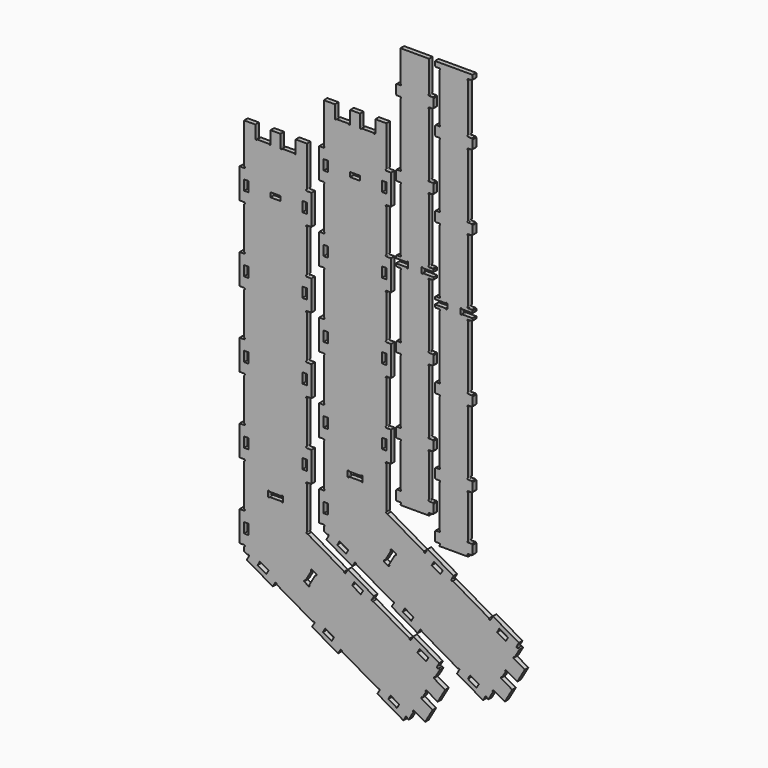
from build123d import *

# Parameters (mm, degrees)
F0_W     = 18.000018
F0_H     = 40.00004
F0_W_2   = 40.00004
F0_H_2   = 18.000018
F1_DEPTH = 18
F2_DEPTH = 18
F3_DEPTH = 18
F4_DEPTH = 18


# Not quite as in the source:
# - ends of sketch curves that miss each other by under 0.0002 mm in the source are joined


with BuildPart() as f1:
    # F0 (on Front) → F1 (new body)
    with BuildSketch(Plane.XZ):
        with BuildLine():
            ThreePointArc((9.416735, 127.137802), (6.159038, 130.277684), (9.166737, 133.657802))
            Line((9.166737, 133.657802), (9.166791, 301.117913))
            ThreePointArc((9.166791, 301.117913), (6.149529, 304.4984), (9.416793, 307.637913))
            Line((9.416793, 307.637913), (27.166753, 307.637922))
            Line((27.166753, 307.637922), (27.166696, 427.138111))
            Line((27.166696, 427.138111), (9.416736, 427.138102))
            ThreePointArc((9.416736, 427.138102), (6.159038, 430.277982), (9.166735, 433.658102))
            Line((9.166735, 433.658102), (9.166735, 601.118252))
            ThreePointArc((9.166735, 601.118252), (6.149472, 604.498738), (9.416735, 607.638252))
            Line((9.416735, 607.638252), (27.166753, 607.638252))
            Line((27.166753, 607.638252), (27.166753, 727.138372))
            Line((27.166753, 727.138372), (9.416735, 727.138372))
            ThreePointArc((9.416735, 727.138372), (6.159037, 730.278253), (9.166735, 733.658372))
            Line((9.166735, 733.658372), (9.166735, 893.835077))
            Line((9.166735, 893.835077), (-35.33331, 893.835077))
            Line((-35.33331, 893.835077), (-35.33331, 844.085027))
            ThreePointArc((-35.33331, 844.085027), (-38.473191, 840.827329), (-41.85331, 843.835027))
            Line((-41.85331, 843.835027), (-89.31337, 843.835027))
            ThreePointArc((-89.31337, 843.835027), (-92.693856, 840.817764), (-95.83337, 844.085027))
            Line((-95.83337, 844.085027), (-95.83337, 893.835077))
            Line((-95.83337, 893.835077), (-135.33341, 893.835077))
            Line((-135.33341, 893.835077), (-135.33341, 844.085027))
            ThreePointArc((-135.33341, 844.085027), (-138.473291, 840.827329), (-141.85341, 843.835027))
            Line((-141.85341, 843.835027), (-189.31347, 843.835027))
            ThreePointArc((-189.31347, 843.835027), (-192.693956, 840.817764), (-195.83347, 844.085027))
            Line((-195.83347, 844.085027), (-195.83347, 893.835077))
            Line((-195.83347, 893.835077), (-240.333515, 893.835077))
            Line((-240.333515, 893.835077), (-240.333515, 733.658372))
            ThreePointArc((-240.333515, 733.658372), (-237.316252, 730.277886), (-240.583515, 727.138372))
            Line((-240.583515, 727.138372), (-258.333533, 727.138372))
            Line((-258.333533, 727.138372), (-258.333533, 607.638252))
            Line((-258.333533, 607.638252), (-240.583515, 607.638252))
            ThreePointArc((-240.583515, 607.638252), (-237.325817, 604.498371), (-240.333515, 601.118252))
            Line((-240.333515, 601.118252), (-240.333515, 433.658102))
            ThreePointArc((-240.333515, 433.658102), (-237.316252, 430.277616), (-240.583515, 427.138102))
            Line((-240.583515, 427.138102), (-258.33359, 427.138093))
            Line((-258.33359, 427.138093), (-258.333533, 307.637922))
            Line((-258.333533, 307.637922), (-240.583457, 307.637931))
            ThreePointArc((-240.583457, 307.637931), (-237.32576, 304.498049), (-240.333459, 301.117931))
            Line((-240.333459, 301.117931), (-240.333513, 133.657802))
            ThreePointArc((-240.333513, 133.657802), (-237.316251, 130.277315), (-240.583515, 127.137802))
            Line((-240.583515, 127.137802), (-258.33359, 127.137793))
            Line((-258.33359, 127.137793), (-258.333533, 7.637622))
            Line((-258.333533, 7.637622), (-240.583457, 7.637631))
            ThreePointArc((-240.583457, 7.637631), (-237.32576, 4.497749), (-240.333459, 1.117631))
            Line((-240.333459, 1.117631), (-240.333513, -166.342498))
            ThreePointArc((-240.333513, -166.342498), (-237.316251, -169.722985), (-240.583515, -172.862498))
            Line((-240.583515, -172.862498), (-258.333591, -172.862507))
            Line((-258.333591, -172.862507), (-258.333533, -292.362678))
            Line((-258.333533, -292.362678), (-240.583457, -292.362669))
            ThreePointArc((-240.583457, -292.362669), (-237.325761, -295.502553), (-240.333461, -298.88267))
            Line((-240.333461, -298.88267), (-240.333555, -466.342558))
            ThreePointArc((-240.333555, -466.342558), (-237.316293, -469.723045), (-240.583558, -472.862558))
            Line((-240.583558, -472.862558), (-258.333576, -472.862609))
            Line((-258.333576, -472.862609), (-258.333634, -592.362729))
            Line((-258.333634, -592.362729), (-240.583616, -592.362738))
            ThreePointArc((-240.583616, -592.362738), (-237.325919, -595.50262), (-240.333619, -598.882738))
            Line((-240.333619, -598.882738), (-240.333626, -614.697808))
            Line((-240.333626, -614.697808), (-226.634429, -622.607044))
            ThreePointArc((-226.634429, -622.607044), (-222.198211, -621.684261), (-221.112943, -626.083551))
            Line((-221.112943, -626.083551), (-229.987952, -641.455517))
            Line((-229.987952, -641.455517), (-126.497812, -701.205577))
            Line((-126.497812, -701.205577), (-117.622803, -685.833611))
            ThreePointArc((-117.622803, -685.833611), (-113.274738, -684.582303), (-111.851318, -688.877104))
            Line((-111.851318, -688.877104), (33.173322, -772.607119))
            ThreePointArc((33.173322, -772.607119), (37.60954, -771.684336), (38.694808, -776.083626))
            Line((38.694808, -776.083626), (29.819778, -791.455646))
            Line((29.819778, -791.455646), (133.309938, -851.205652))
            Line((133.309938, -851.205652), (142.184969, -835.833632))
            ThreePointArc((142.184969, -835.833632), (146.533035, -834.582325), (147.956454, -838.877127))
            Line((147.956454, -838.877127), (292.98123, -922.607283))
            ThreePointArc((292.98123, -922.607283), (297.417448, -921.684501), (298.502715, -926.083791))
            Line((298.502715, -926.083791), (289.627706, -941.455757))
            Line((289.627706, -941.455757), (393.117846, -1001.205817))
            Line((393.117846, -1001.205817), (401.992855, -985.833851))
            ThreePointArc((401.992855, -985.833851), (406.34092, -984.582543), (407.76434, -988.877344))
            Line((407.76434, -988.877344), (413.640981, -992.270225))
            Line((413.640981, -992.270225), (432.880981, -958.945543))
            ThreePointArc((432.880981, -958.945543), (431.958197, -954.509325), (436.357486, -953.424056))
            Line((436.357486, -953.424056), (479.442305, -978.299088))
            Line((479.442305, -978.299088), (509.193048, -926.76929))
            Line((509.193048, -926.76929), (466.108229, -901.894258))
            ThreePointArc((466.108229, -901.894258), (464.85692, -897.546192), (469.151722, -896.122772))
            Line((469.151722, -896.122772), (482.881029, -872.342915))
            ThreePointArc((482.881029, -872.342915), (481.958246, -867.906697), (486.357536, -866.821429))
            Line((486.357536, -866.821429), (529.442343, -891.696454))
            Line((529.442343, -891.696454), (559.192373, -840.167891))
            Line((559.192373, -840.167891), (516.107566, -815.292866))
            ThreePointArc((516.107566, -815.292866), (514.856259, -810.9448), (519.151061, -809.521381))
            Line((519.151061, -809.521381), (538.391794, -776.195479))
            Line((538.391794, -776.195479), (532.514818, -772.803231))
            ThreePointArc((532.514818, -772.803231), (528.078695, -773.726473), (526.992973, -769.327295))
            Line((526.992973, -769.327295), (535.867989, -753.955317))
            Line((535.867989, -753.955317), (432.377849, -694.205257))
            Line((432.377849, -694.205257), (423.50284, -709.577223))
            ThreePointArc((423.50284, -709.577223), (419.154774, -710.828532), (417.731354, -706.53373))
            Line((417.731354, -706.53373), (272.70661, -622.803654))
            ThreePointArc((272.70661, -622.803654), (268.270393, -623.726438), (267.185125, -619.327148))
            Line((267.185125, -619.327148), (276.060155, -603.955127))
            Line((276.060155, -603.955127), (172.569942, -544.205091))
            Line((172.569942, -544.205091), (163.694912, -559.577112))
            ThreePointArc((163.694912, -559.577112), (159.346846, -560.828419), (157.923427, -556.533617))
            Line((157.923427, -556.533617), (12.426692, -472.530975))
            ThreePointArc((12.426692, -472.530975), (8.095684, -471.267159), (9.166694, -466.884489))
            Line((9.166694, -466.884489), (9.166734, -298.882678))
            ThreePointArc((9.166734, -298.882678), (6.149471, -295.502192), (9.416735, -292.362678))
            Line((9.416735, -292.362678), (27.166811, -292.36267))
            Line((27.166811, -292.36267), (27.166754, -172.862558))
            Line((27.166754, -172.862558), (9.416678, -172.862567))
            ThreePointArc((9.416678, -172.862567), (6.158982, -169.722684), (9.166682, -166.342567))
            Line((9.166682, -166.342567), (9.166789, 1.117613))
            ThreePointArc((9.166789, 1.117613), (6.149528, 4.498101), (9.416793, 7.637613))
            Line((9.416793, 7.637613), (27.166753, 7.637622))
            Line((27.166753, 7.637622), (27.166696, 127.137811))
            Line((27.166696, 127.137811), (9.416735, 127.137802))
        make_face()
        Polygon((-186.688399, -645.958571), (-177.68839, -630.370098), (-143.047339, -650.370118), (-152.047348, -665.958591), align=None, mode=Mode.SUBTRACT)
        Polygon((-240.583577, -512.612658), (-222.583559, -512.612667), (-222.583579, -552.612707), (-240.583597, -552.612698), align=None, mode=Mode.SUBTRACT)
        with BuildLine():
            ThreePointArc((-91.850917, -373.359332), (-88.471691, -370.34449), (-85.333339, -373.609331))
            Line((-85.333339, -373.609331), (-85.333344, -391.609218))
            ThreePointArc((-85.333344, -391.609218), (-88.471971, -394.866907), (-91.850922, -391.859215))
            Line((-91.850922, -391.859215), (-139.315866, -391.85919))
            ThreePointArc((-139.315866, -391.85919), (-142.695093, -394.87403), (-145.833443, -391.609186))
            Line((-145.833443, -391.609186), (-145.833431, -373.609343))
            ThreePointArc((-145.833431, -373.609343), (-142.694806, -370.351652), (-139.315853, -373.359342))
            Line((-139.315853, -373.359342), (-91.850917, -373.359332))
        make_face(mode=Mode.SUBTRACT)
        Polygon((-240.583534, -212.612607), (-222.583497, -212.612598), (-222.583478, -252.612629), (-240.583515, -252.612638), align=None, mode=Mode.SUBTRACT)
        Polygon((73.119352, -795.958646), (82.119344, -780.370185), (116.760412, -800.370193), (107.76042, -815.958653), align=None, mode=Mode.SUBTRACT)
        with BuildLine():
            ThreePointArc((26.891612, -597.527447), (25.970296, -593.093531), (30.366907, -592.00806))
            Line((30.366907, -592.00806), (45.958208, -601.009702))
            ThreePointArc((45.958208, -601.009702), (47.210138, -605.356677), (42.915926, -606.77909))
            Line((42.915926, -606.77909), (19.183457, -647.884929))
            ThreePointArc((19.183457, -647.884929), (20.104773, -652.318846), (15.708162, -653.404317))
            Line((15.708162, -653.404317), (0.116861, -644.402675))
            ThreePointArc((0.116861, -644.402675), (-1.135069, -640.0557), (3.159143, -638.633287))
            Line((3.159143, -638.633287), (26.891612, -597.527447))
        make_face(mode=Mode.SUBTRACT)
        Polygon((332.927259, -945.958811), (341.927268, -930.370338), (376.568319, -950.370358), (367.56831, -965.958831), align=None, mode=Mode.SUBTRACT)
        Polygon((448.927375, -745.040716), (457.927384, -729.452243), (492.568435, -749.452263), (483.568426, -765.040736), align=None, mode=Mode.SUBTRACT)
        Polygon((189.119467, -595.040572), (198.119478, -579.452078), (232.760531, -599.452077), (223.760519, -615.040571), align=None, mode=Mode.SUBTRACT)
        Polygon((-8.583263, -252.612647), (-8.583283, -212.612598), (9.416716, -212.612589), (9.416735, -252.612638), align=None, mode=Mode.SUBTRACT)
        Polygon((-222.583516, 87.387771), (-222.583497, 47.387722), (-240.583496, 47.387713), (-240.583515, 87.387762), align=None, mode=Mode.SUBTRACT)
        Polygon((-222.583516, 387.388071), (-222.583497, 347.388022), (-240.583496, 347.388013), (-240.583515, 387.388062), align=None, mode=Mode.SUBTRACT)
        with Locations((-231.583506, 667.388312)):
            Rectangle(F0_W, F0_H, mode=Mode.SUBTRACT)
        with Locations((-115.583419, 667.38811)):
            Rectangle(F0_W_2, F0_H_2, mode=Mode.SUBTRACT)
        Polygon((9.416735, 47.387722), (-8.583263, 47.387713), (-8.583283, 87.387762), (9.416716, 87.387771), align=None, mode=Mode.SUBTRACT)
        Polygon((9.416735, 347.388022), (-8.583263, 347.388013), (-8.583283, 387.388062), (9.416716, 387.388071), align=None, mode=Mode.SUBTRACT)
        with Locations((0.416726, 667.388312)):
            Rectangle(F0_W, F0_H, mode=Mode.SUBTRACT)
    extrude(amount=F1_DEPTH)


with BuildPart() as f2:
    # F0 (on Front) → F2 (new body)
    with BuildSketch(Plane.XZ):
        with BuildLine():
            Line((178.620772, 1175.027534), (64.620346, 1175.026565))
            Line((64.620346, 1175.026565), (64.621399, 1051.046435))
            ThreePointArc((64.621399, 1051.046435), (67.631425, 1048.03646), (64.62145, 1045.026435))
            Line((64.62145, 1045.026435), (49.621435, 1045.026002))
            Line((49.621435, 1045.026002), (46.621458, 1042.026279))
            Line((46.621458, 1042.026279), (46.621747, 1008.026245))
            Line((46.621747, 1008.026245), (49.621775, 1005.025962))
            Line((49.621775, 1005.025962), (64.62179, 1005.02609))
            ThreePointArc((64.62179, 1005.02609), (67.631845, 1002.016145), (64.6219, 999.00609))
            Line((64.6219, 999.00609), (64.626436, 751.046135))
            ThreePointArc((64.626436, 751.046135), (67.636491, 748.03619), (64.626546, 745.026135))
            Line((64.626546, 745.026135), (49.626531, 745.025702))
            Line((49.626531, 745.025702), (46.626554, 742.025979))
            Line((46.626554, 742.025979), (46.626843, 708.025945))
            Line((46.626843, 708.025945), (49.626871, 705.025662))
            Line((49.626871, 705.025662), (64.626886, 705.02579))
            ThreePointArc((64.626886, 705.02579), (67.636927, 702.01583), (64.626967, 699.00579))
            Line((64.626967, 699.00579), (64.630288, 451.044593))
            ThreePointArc((64.630288, 451.044593), (67.640328, 448.034634), (64.630369, 445.024593))
            Line((64.630369, 445.024593), (49.630354, 445.024466))
            Line((49.630354, 445.024466), (46.630376, 442.024743))
            Line((46.630376, 442.024743), (46.62917, 434.024429))
            Line((46.62917, 434.024429), (89.609219, 434.025159))
            ThreePointArc((89.609219, 434.025159), (92.619168, 437.03521), (95.629219, 434.025262))
            Line((95.629219, 434.025262), (95.629525, 416.025244))
            ThreePointArc((95.629525, 416.025244), (92.619577, 413.015193), (89.609525, 416.025141))
            Line((89.609525, 416.025141), (46.629476, 416.024411))
            Line((46.629476, 416.024411), (46.630665, 408.024403))
            Line((46.630665, 408.024403), (49.630693, 405.024426))
            Line((49.630693, 405.024426), (64.630708, 405.024553))
            ThreePointArc((64.630708, 405.024553), (67.640778, 402.014623), (64.630848, 399.004553))
            Line((64.630848, 399.004553), (64.636599, 151.045536))
            ThreePointArc((64.636599, 151.045536), (67.646669, 148.035606), (64.636739, 145.025536))
            Line((64.636739, 145.025536), (49.636724, 145.025102))
            Line((49.636724, 145.025102), (46.636746, 142.02538))
            Line((46.636746, 142.02538), (46.637035, 108.025346))
            Line((46.637035, 108.025346), (49.637064, 105.025062))
            Line((49.637064, 105.025062), (64.637079, 105.02519))
            ThreePointArc((64.637079, 105.02519), (67.647134, 102.015245), (64.637189, 99.00519))
            Line((64.637189, 99.00519), (64.641725, -148.954764))
            ThreePointArc((64.641725, -148.954764), (67.65178, -151.964709), (64.641835, -154.974764))
            Line((64.641835, -154.974764), (49.64182, -154.975198))
            Line((49.64182, -154.975198), (46.641842, -157.97492))
            Line((46.641842, -157.97492), (46.642131, -191.974954))
            Line((46.642131, -191.974954), (49.64216, -194.975238))
            Line((49.64216, -194.975238), (64.642175, -194.97511))
            ThreePointArc((64.642175, -194.97511), (67.652243, -197.985042), (64.64231, -200.99511))
            Line((64.64231, -200.99511), (64.646081, -368.954984))
            ThreePointArc((64.646081, -368.954984), (67.656148, -371.964916), (64.646216, -374.974984))
            Line((64.646216, -374.974984), (49.646201, -374.975417))
            Line((49.646201, -374.975417), (46.646224, -377.97514))
            Line((46.646224, -377.97514), (46.646512, -411.975174))
            Line((46.646512, -411.975174), (49.646541, -414.975457))
            Line((49.646541, -414.975457), (64.646556, -414.97533))
            ThreePointArc((64.646556, -414.97533), (67.656634, -417.985253), (64.646711, -420.99533))
            Line((64.646711, -420.99533), (64.646808, -424.739202))
            Line((64.646808, -424.739202), (178.647234, -424.739202))
            Line((178.647234, -424.739202), (178.647137, -420.994362))
            ThreePointArc((178.647137, -420.994362), (175.637059, -417.98444), (178.646981, -414.974362))
            Line((178.646981, -414.974362), (193.646996, -414.974234))
            Line((193.646996, -414.974234), (196.646974, -411.974206))
            Line((196.646974, -411.974206), (196.646685, -377.974172))
            Line((196.646685, -377.974172), (193.646657, -374.974194))
            Line((193.646657, -374.974194), (178.646642, -374.974016))
            ThreePointArc((178.646642, -374.974016), (175.636574, -371.964084), (178.646506, -368.954016))
            Line((178.646506, -368.954016), (178.642735, -200.994142))
            ThreePointArc((178.642735, -200.994142), (175.632667, -197.98421), (178.6426, -194.974142))
            Line((178.6426, -194.974142), (193.642615, -194.974014))
            Line((193.642615, -194.974014), (196.642593, -191.973986))
            Line((196.642593, -191.973986), (196.642304, -157.973952))
            Line((196.642304, -157.973952), (193.642276, -154.973974))
            Line((193.642276, -154.973974), (178.642261, -154.973796))
            ThreePointArc((178.642261, -154.973796), (175.632205, -151.963852), (178.64215, -148.953796))
            Line((178.64215, -148.953796), (178.637614, 99.006158))
            ThreePointArc((178.637614, 99.006158), (175.627559, 102.016103), (178.637504, 105.026158))
            Line((178.637504, 105.026158), (193.637519, 105.026285))
            Line((193.637519, 105.026285), (196.637497, 108.026314))
            Line((196.637497, 108.026314), (196.637208, 142.026348))
            Line((196.637208, 142.026348), (193.637179, 145.026325))
            Line((193.637179, 145.026325), (178.637164, 145.026504))
            ThreePointArc((178.637164, 145.026504), (175.627095, 148.036434), (178.637025, 151.046504))
            Line((178.637025, 151.046504), (178.631274, 399.005521))
            ThreePointArc((178.631274, 399.005521), (175.621204, 402.015451), (178.631134, 405.025521))
            Line((178.631134, 405.025521), (193.631149, 405.025649))
            Line((193.631149, 405.025649), (196.631126, 408.025677))
            Line((196.631126, 408.025677), (196.628594, 416.026959))
            Line((196.628594, 416.026959), (153.648545, 416.026229))
            ThreePointArc((153.648545, 416.026229), (150.638596, 413.016178), (147.628545, 416.026127))
            Line((147.628545, 416.026127), (147.628239, 434.026145))
            ThreePointArc((147.628239, 434.026145), (150.638188, 437.036196), (153.648239, 434.026247))
            Line((153.648239, 434.026247), (196.628288, 434.026977))
            Line((196.628288, 434.026977), (196.630838, 442.026017))
            Line((196.630838, 442.026017), (193.630809, 445.025995))
            Line((193.630809, 445.025995), (178.630794, 445.025561))
            ThreePointArc((178.630794, 445.025561), (175.620754, 448.035521), (178.630714, 451.045561))
            Line((178.630714, 451.045561), (178.627392, 699.006758))
            ThreePointArc((178.627392, 699.006758), (175.617352, 702.016718), (178.627312, 705.026758))
            Line((178.627312, 705.026758), (193.627327, 705.026885))
            Line((193.627327, 705.026885), (196.627304, 708.026914))
            Line((196.627304, 708.026914), (196.627016, 742.026948))
            Line((196.627016, 742.026948), (193.626987, 745.026925))
            Line((193.626987, 745.026925), (178.626972, 745.027104))
            ThreePointArc((178.626972, 745.027104), (175.616917, 748.037049), (178.626862, 751.047104))
            Line((178.626862, 751.047104), (178.622326, 999.007058))
            ThreePointArc((178.622326, 999.007058), (175.612271, 1002.017003), (178.622216, 1005.027058))
            Line((178.622216, 1005.027058), (193.622231, 1005.027185))
            Line((193.622231, 1005.027185), (196.622208, 1008.027214))
            Line((196.622208, 1008.027214), (196.621919, 1042.027248))
            Line((196.621919, 1042.027248), (193.621891, 1045.027225))
            Line((193.621891, 1045.027225), (178.621876, 1045.027404))
            ThreePointArc((178.621876, 1045.027404), (175.611851, 1048.037379), (178.621825, 1051.047404))
            Line((178.621825, 1051.047404), (178.620772, 1175.027534))
        make_face()
        Polygon((135.824732, 535.317923), (135.827154, 534.955858), (135.830132, 534.588475), (135.823797, 534.221876), (135.808216, 533.856229), (135.783454, 533.491705), (135.749579, 533.12847), (135.706655, 532.766695), (135.654751, 532.406547), (135.59393, 532.048196), (135.524261, 531.69181), (135.445809, 531.337559), (135.35864, 530.98561), (135.26282, 530.636133), (135.158417, 530.289296), (135.045495, 529.945269), (134.924122, 529.604219), (134.794363, 529.266316), (134.656284, 528.931728), (134.509953, 528.600625), (134.355434, 528.273174), (134.192796, 527.949546), (134.022102, 527.629907), (133.84342, 527.314428), (133.656817, 527.003277), (133.462357, 526.696623), (133.260108, 526.394635), (133.050136, 526.09748), (132.832507, 525.805329), (132.607286, 525.518349), (132.374541, 525.23671), (132.134338, 524.960581), (131.886742, 524.690129), (131.631821, 524.425524), (131.299075, 524.119397), (130.95941, 523.822315), (130.613032, 523.534359), (130.260144, 523.255604), (129.900953, 522.986129), (129.535661, 522.726011), (129.164474, 522.475329), (128.787597, 522.23416), (128.405234, 522.002581), (128.01759, 521.780672), (127.624869, 521.568508), (127.227276, 521.366169), (126.825016, 521.173731), (126.418293, 520.991273), (126.007313, 520.818873), (125.592279, 520.656608), (125.173397, 520.504555), (124.75087, 520.362793), (124.324905, 520.2314), (123.895704, 520.110453), (123.463474, 520.000029), (123.028418, 519.900208), (122.590742, 519.811066), (122.150649, 519.732681), (121.708345, 519.66513), (121.264034, 519.608493), (120.817921, 519.562846), (120.370211, 519.528268), (119.921108, 519.504835), (119.470816, 519.492626), (119.019541, 519.491719), (118.567488, 519.502191), (118.076507, 519.488129), (117.586341, 519.486573), (117.097216, 519.497438), (116.609361, 519.520639), (116.123, 519.556089), (115.638362, 519.603705), (115.155673, 519.663399), (114.675159, 519.735087), (114.197049, 519.818683), (113.721568, 519.914102), (113.248944, 520.021258), (112.779404, 520.140066), (112.313173, 520.27044), (111.85048, 520.412296), (111.391551, 520.565547), (110.936613, 520.730108), (110.485892, 520.905893), (110.039616, 521.092818), (109.598012, 521.290796), (109.161306, 521.499743), (108.729725, 521.719573), (108.303497, 521.950199), (107.882847, 522.191538), (107.468003, 522.443503), (107.059192, 522.70601), (106.656641, 522.978972), (106.260576, 523.262303), (105.871224, 523.55592), (105.488812, 523.859736), (105.113568, 524.173666), (104.745717, 524.497623), (104.385488, 524.831524), (104.131148, 525.081554), (103.883989, 525.337593), (103.644082, 525.599468), (103.411499, 525.867009), (103.18631, 526.140045), (102.968587, 526.418403), (102.758402, 526.701914), (102.555826, 526.990404), (102.36093, 527.283704), (102.173785, 527.581642), (101.994464, 527.884046), (101.823036, 528.190745), (101.659575, 528.501568), (101.50415, 528.816343), (101.356833, 529.1349), (101.217696, 529.457066), (101.08681, 529.782671), (100.964246, 530.111543), (100.850076, 530.44351), (100.744371, 530.778403), (100.647202, 531.116048), (100.558641, 531.456275), (100.47876, 531.798913), (100.407628, 532.14379), (100.345319, 532.490735), (100.291902, 532.839576), (100.24745, 533.190143), (100.212034, 533.542263), (100.185725, 533.895766), (100.168594, 534.250481), (100.160714, 534.606235), (100.162154, 534.962858), (100.165368, 535.325325), (100.178024, 535.686798), (100.200048, 536.047104), (100.231366, 536.40607), (100.271903, 536.763521), (100.321587, 537.119285), (100.380343, 537.473187), (100.448097, 537.825056), (100.524775, 538.174716), (100.610304, 538.521994), (100.704609, 538.866718), (100.807617, 539.208713), (100.919254, 539.547806), (101.039445, 539.883825), (101.168117, 540.216594), (101.305196, 540.545941), (101.450608, 540.871692), (101.604279, 541.193674), (101.766135, 541.511714), (101.936103, 541.825638), (102.114108, 542.135271), (102.300076, 542.440442), (102.493934, 542.740977), (102.695607, 543.036701), (102.905023, 543.327442), (103.122105, 543.613027), (103.346782, 543.893281), (103.578979, 544.168031), (103.818622, 544.437104), (104.065637, 544.700326), (104.31995, 544.957524), (104.581488, 545.208524), (104.939825, 545.532432), (105.3055, 545.846538), (105.678293, 546.150763), (106.057982, 546.445027), (106.444344, 546.729248), (106.837157, 547.003348), (107.236201, 547.267244), (107.641253, 547.520858), (108.052092, 547.764108), (108.468496, 547.996915), (108.890242, 548.219197), (109.317111, 548.430876), (109.748878, 548.63187), (110.185324, 548.822099), (110.626226, 549.001483), (111.071363, 549.169941), (111.520512, 549.327393), (111.973452, 549.47376), (112.429961, 549.608959), (112.889818, 549.732912), (113.3528, 549.845538), (113.818687, 549.946756), (114.287255, 550.036487), (114.758284, 550.114649), (115.231552, 550.181163), (115.706837, 550.235948), (116.183918, 550.278925), (116.662572, 550.310011), (117.142577, 550.329128), (117.623713, 550.336195), (118.105757, 550.331132), (118.588488, 550.313858), (119.038962, 550.321233), (119.488559, 550.317164), (119.937072, 550.30173), (120.384293, 550.275011), (120.830015, 550.237089), (121.274032, 550.188042), (121.716135, 550.127952), (122.156118, 550.056899), (122.593773, 549.974963), (123.028893, 549.882225), (123.461271, 549.778765), (123.8907, 549.664662), (124.316973, 549.539998), (124.739882, 549.404853), (125.15922, 549.259307), (125.574779, 549.103441), (125.986354, 548.937334), (126.393735, 548.761068), (126.796717, 548.574721), (127.195092, 548.378376), (127.588653, 548.172111), (127.977193, 547.956008), (128.360503, 547.730147), (128.738378, 547.494608), (129.11061, 547.249471), (129.476992, 546.994816), (129.837316, 546.730725), (130.191375, 546.457277), (130.538962, 546.174552), (130.879871, 545.882632), (131.213893, 545.581596), (131.540821, 545.271524), (131.795633, 545.014356), (132.043335, 544.751337), (132.283858, 544.482632), (132.517134, 544.208404), (132.743094, 543.928818), (132.961669, 543.64404), (133.17279, 543.354232), (133.376389, 543.059561), (133.572396, 542.760189), (133.760743, 542.456283), (133.941362, 542.148006), (134.114182, 541.835522), (134.279136, 541.518997), (134.436155, 541.198595), (134.58517, 540.874479), (134.726113, 540.546816), (134.858913, 540.215769), (134.983503, 539.881502), (135.099814, 539.544181), (135.207777, 539.203969), (135.307324, 538.861031), (135.398384, 538.515532), (135.480891, 538.167637), (135.554774, 537.817509), (135.619965, 537.465313), (135.676396, 537.111213), (135.723997, 536.755375), (135.7627, 536.397962), (135.792436, 536.03914), (135.813137, 535.679072), align=None, mode=Mode.SUBTRACT)
        Polygon((135.824732, 574.03259), (135.827154, 573.670524), (135.830132, 573.303141), (135.823797, 572.936542), (135.808216, 572.570896), (135.783454, 572.206371), (135.749579, 571.843137), (135.706655, 571.481361), (135.654751, 571.121214), (135.59393, 570.762863), (135.524261, 570.406477), (135.445809, 570.052226), (135.35864, 569.700277), (135.26282, 569.3508), (135.158417, 569.003963), (135.045495, 568.659935), (134.924122, 568.318886), (134.794363, 567.980983), (134.656284, 567.646395), (134.509953, 567.315292), (134.355434, 566.987841), (134.192796, 566.664212), (134.022102, 566.344574), (133.84342, 566.029095), (133.656817, 565.717944), (133.462357, 565.41129), (133.260108, 565.109301), (133.050136, 564.812147), (132.832507, 564.519995), (132.607286, 564.233016), (132.374541, 563.951377), (132.134338, 563.675247), (131.886742, 563.404796), (131.631821, 563.140191), (131.299075, 562.834063), (130.95941, 562.536982), (130.613032, 562.249025), (130.260144, 561.97027), (129.900953, 561.700795), (129.535661, 561.440678), (129.164474, 561.189996), (128.787597, 560.948826), (128.405234, 560.717248), (128.01759, 560.495338), (127.624869, 560.283175), (127.227276, 560.080835), (126.825016, 559.888398), (126.418293, 559.70594), (126.007313, 559.53354), (125.592279, 559.371274), (125.173397, 559.219222), (124.75087, 559.07746), (124.324905, 558.946067), (123.895704, 558.825119), (123.463474, 558.714696), (123.028418, 558.614874), (122.590742, 558.525732), (122.150649, 558.447347), (121.708345, 558.379797), (121.264034, 558.32316), (120.817921, 558.277513), (120.370211, 558.242934), (119.921108, 558.219502), (119.470816, 558.207293), (119.019541, 558.206386), (118.567488, 558.216858), (118.076507, 558.202796), (117.586341, 558.20124), (117.097216, 558.212105), (116.609361, 558.235306), (116.123, 558.270756), (115.638362, 558.318371), (115.155673, 558.378066), (114.675159, 558.449753), (114.197049, 558.53335), (113.721568, 558.628768), (113.248944, 558.735925), (112.779404, 558.854733), (112.313173, 558.985107), (111.85048, 559.126962), (111.391551, 559.280213), (110.936613, 559.444774), (110.485892, 559.62056), (110.039616, 559.807485), (109.598012, 560.005463), (109.161306, 560.21441), (108.729725, 560.434239), (108.303497, 560.664866), (107.882847, 560.906205), (107.468003, 561.15817), (107.059192, 561.420676), (106.656641, 561.693638), (106.260576, 561.97697), (105.871224, 562.270587), (105.488812, 562.574403), (105.113568, 562.888332), (104.745717, 563.21229), (104.385488, 563.546191), (104.131148, 563.796221), (103.883989, 564.052259), (103.644082, 564.314135), (103.411499, 564.581676), (103.18631, 564.854711), (102.968587, 565.13307), (102.758402, 565.41658), (102.555826, 565.705071), (102.36093, 565.998371), (102.173785, 566.296309), (101.994464, 566.598713), (101.823036, 566.905412), (101.659575, 567.216235), (101.50415, 567.53101), (101.356833, 567.849566), (101.217696, 568.171733), (101.08681, 568.497337), (100.964246, 568.826209), (100.850076, 569.158177), (100.744371, 569.493069), (100.647202, 569.830715), (100.558641, 570.170942), (100.47876, 570.51358), (100.407628, 570.858457), (100.345319, 571.205401), (100.291902, 571.554243), (100.24745, 571.904809), (100.212034, 572.25693), (100.185725, 572.610433), (100.168594, 572.965147), (100.160714, 573.320901), (100.162154, 573.677524), (100.165368, 574.039991), (100.178024, 574.401465), (100.200048, 574.761771), (100.231366, 575.120737), (100.271903, 575.478188), (100.321587, 575.833952), (100.380343, 576.187854), (100.448097, 576.539722), (100.524775, 576.889382), (100.610304, 577.236661), (100.704609, 577.581384), (100.807617, 577.92338), (100.919254, 578.262473), (101.039445, 578.598491), (101.168117, 578.931261), (101.305196, 579.260608), (101.450608, 579.586359), (101.604279, 579.908341), (101.766135, 580.226381), (101.936103, 580.540304), (102.114108, 580.849938), (102.300076, 581.155109), (102.493934, 581.455644), (102.695607, 581.751368), (102.905023, 582.042109), (103.122105, 582.327693), (103.346782, 582.607947), (103.578979, 582.882697), (103.818622, 583.15177), (104.065637, 583.414993), (104.31995, 583.672191), (104.581488, 583.923191), (104.939825, 584.247098), (105.3055, 584.561205), (105.678293, 584.86543), (106.057982, 585.159694), (106.444344, 585.443915), (106.837157, 585.718014), (107.236201, 585.981911), (107.641253, 586.235524), (108.052092, 586.478775), (108.468496, 586.711581), (108.890242, 586.933864), (109.317111, 587.145542), (109.748878, 587.346536), (110.185324, 587.536765), (110.626226, 587.716149), (111.071363, 587.884608), (111.520512, 588.04206), (111.973452, 588.188426), (112.429961, 588.323626), (112.889818, 588.447579), (113.3528, 588.560205), (113.818687, 588.661423), (114.287255, 588.751154), (114.758284, 588.829316), (115.231552, 588.89583), (115.706837, 588.950615), (116.183918, 588.993591), (116.662572, 589.024678), (117.142577, 589.043795), (117.623713, 589.050862), (118.105757, 589.045798), (118.588488, 589.028524), (119.038962, 589.0359), (119.488559, 589.031831), (119.937072, 589.016396), (120.384293, 588.989678), (120.830015, 588.951755), (121.274032, 588.902709), (121.716135, 588.842619), (122.156118, 588.771566), (122.593773, 588.68963), (123.028893, 588.596892), (123.461271, 588.493431), (123.8907, 588.379329), (124.316973, 588.254665), (124.739882, 588.11952), (125.15922, 587.973974), (125.574779, 587.818108), (125.986354, 587.652001), (126.393735, 587.475734), (126.796717, 587.289388), (127.195092, 587.093042), (127.588653, 586.886778), (127.977193, 586.670675), (128.360503, 586.444814), (128.738378, 586.209274), (129.11061, 585.964137), (129.476992, 585.709483), (129.837316, 585.445392), (130.191375, 585.171944), (130.538962, 584.889219), (130.879871, 584.597299), (131.213893, 584.296263), (131.540821, 583.986191), (131.795633, 583.729023), (132.043335, 583.466004), (132.283858, 583.197298), (132.517134, 582.92307), (132.743094, 582.643485), (132.961669, 582.358706), (133.17279, 582.068899), (133.376389, 581.774227), (133.572396, 581.474856), (133.760743, 581.17095), (133.941362, 580.862672), (134.114182, 580.550189), (134.279136, 580.233664), (134.436155, 579.913261), (134.58517, 579.589146), (134.726113, 579.261483), (134.858913, 578.930435), (134.983503, 578.596169), (135.099814, 578.258847), (135.207777, 577.918636), (135.307324, 577.575698), (135.398384, 577.230199), (135.480891, 576.882303), (135.554774, 576.532175), (135.619965, 576.179979), (135.676396, 575.82588), (135.723997, 575.470042), (135.7627, 575.112629), (135.792436, 574.753807), (135.813137, 574.393739), align=None, mode=Mode.SUBTRACT)
        Polygon((117.846488, 612.287191), (117.846488, 596.924524), (100.372154, 596.924524), (100.372154, 612.287191), (100.375132, 612.71977), (100.400464, 613.149836), (100.447808, 613.576574), (100.516821, 613.999165), (100.607162, 614.416793), (100.71849, 614.828642), (100.850462, 615.233894), (101.002738, 615.631733), (101.174974, 616.021341), (101.366829, 616.401901), (101.577961, 616.772598), (101.808029, 617.132613), (102.056691, 617.48113), (102.323605, 617.817332), (102.608429, 618.140403), (102.910821, 618.449524), (103.21839, 618.747408), (103.539454, 619.028346), (103.873232, 619.292016), (104.218946, 619.538097), (104.575816, 619.766268), (104.943063, 619.976208), (105.319908, 620.167595), (105.705571, 620.340108), (106.099273, 620.493425), (106.500235, 620.627226), (106.907677, 620.741189), (107.320821, 620.834993), (107.738886, 620.908316), (108.161094, 620.960838), (108.586666, 620.992237), (109.014821, 621.002191), (109.453687, 621.004789), (109.890359, 620.984805), (110.324009, 620.94257), (110.75381, 620.878415), (111.178936, 620.792672), (111.598559, 620.685673), (112.011852, 620.55775), (112.417988, 620.409233), (112.816139, 620.240454), (113.205478, 620.051745), (113.585179, 619.843437), (113.954415, 619.615863), (114.312357, 619.369353), (114.658179, 619.104238), (114.991054, 618.820852), (115.310154, 618.519524), (115.611264, 618.204413), (115.894878, 617.875615), (116.16067, 617.533939), (116.408316, 617.180191), (116.637491, 616.815177), (116.847871, 616.439704), (117.039131, 616.054579), (117.210946, 615.660608), (117.362991, 615.258598), (117.494943, 614.849355), (117.606475, 614.433687), (117.697264, 614.012399), (117.766984, 613.586299), (117.815311, 613.156194), (117.841921, 612.722889), align=None, mode=Mode.SUBTRACT)
        Polygon((135.753889, 672.61038), (135.771154, 672.095191), (135.772177, 671.579978), (135.746631, 671.06749), (135.694911, 670.558699), (135.617409, 670.054582), (135.514519, 669.55611), (135.386633, 669.064259), (135.234144, 668.580003), (135.057446, 668.104316), (134.856931, 667.638172), (134.632993, 667.182544), (134.386025, 666.738408), (134.11642, 666.306738), (133.82457, 665.888507), (133.51087, 665.484689), (133.175711, 665.096259), (132.819488, 664.724191), (132.563259, 664.466058), (132.300879, 664.215393), (132.032527, 663.972271), (131.758381, 663.736763), (131.478622, 663.508941), (131.193428, 663.28888), (130.902978, 663.076651), (130.607451, 662.872326), (130.307026, 662.67598), (130.001882, 662.487683), (129.692198, 662.307509), (129.378154, 662.135531), (129.059927, 661.97182), (128.737697, 661.816451), (128.411644, 661.669495), (128.081946, 661.531024), (127.748782, 661.401113), (127.412331, 661.279832), (127.072772, 661.167255), (126.730285, 661.063455), (126.385048, 660.968504), (126.03724, 660.882475), (125.68704, 660.80544), (125.334628, 660.737472), (124.980182, 660.678644), (124.623882, 660.629028), (124.265905, 660.588697), (123.906432, 660.557723), (123.545642, 660.53618), (123.183712, 660.52414), (122.820824, 660.521675), (122.457154, 660.528858), (122.095088, 660.514807), (121.733499, 660.509803), (121.372548, 660.513788), (121.012397, 660.526702), (120.653208, 660.548488), (120.295144, 660.579086), (119.938365, 660.618439), (119.583034, 660.666488), (119.229314, 660.723174), (118.877365, 660.788438), (118.527349, 660.862223), (118.17943, 660.944469), (117.833768, 661.035118), (117.490525, 661.134112), (117.149864, 661.241392), (116.811946, 661.356899), (116.476933, 661.480576), (116.144988, 661.612362), (115.816272, 661.752201), (115.490947, 661.900033), (115.169174, 662.055799), (114.851117, 662.219442), (114.536937, 662.390903), (114.226795, 662.570123), (113.920854, 662.757044), (113.619275, 662.951607), (113.322222, 663.153753), (113.029854, 663.363425), (112.742335, 663.580563), (112.459826, 663.805109), (112.18249, 664.037004), (111.910488, 664.276191), (111.546329, 664.678951), (111.203096, 665.097378), (110.881149, 665.530572), (110.580852, 665.977628), (110.302567, 666.437646), (110.046656, 666.909722), (109.813481, 667.392955), (109.603404, 667.886441), (109.416789, 668.389279), (109.253997, 668.900566), (109.11539, 669.4194), (109.001331, 669.944878), (108.912183, 670.476099), (108.848307, 671.01216), (108.810065, 671.552158), (108.797821, 672.095191), (108.823224, 672.62103), (108.876361, 673.142607), (108.956746, 673.658886), (109.063894, 674.168832), (109.197319, 674.671408), (109.356536, 675.16558), (109.541059, 675.650311), (109.750404, 676.124566), (109.984085, 676.587309), (110.241616, 677.037505), (110.522513, 677.474118), (110.82629, 677.896113), (111.152461, 678.302453), (111.500541, 678.692103), (111.870045, 679.064028), (112.260488, 679.417191), (112.518645, 679.657429), (112.78244, 679.89029), (113.051698, 680.115708), (113.326247, 680.333621), (113.605912, 680.543965), (113.89052, 680.746677), (114.179898, 680.941691), (114.473873, 681.128946), (114.77227, 681.308377), (115.074917, 681.479921), (115.38164, 681.643513), (115.692265, 681.799091), (116.006619, 681.946591), (116.324529, 682.085948), (116.645821, 682.2171), (116.970321, 682.339983), (117.297856, 682.454532), (117.628254, 682.560685), (117.961339, 682.658377), (118.296939, 682.747546), (118.634881, 682.828127), (118.97499, 682.900056), (119.317094, 682.963271), (119.661019, 683.017707), (120.006591, 683.0633), (120.353637, 683.099988), (120.701984, 683.127706), (121.051458, 683.146391), (121.401885, 683.155979), (121.753093, 683.156406), (122.104907, 683.147609), (122.457154, 683.129524), (122.806929, 683.141224), (123.156145, 683.143987), (123.504639, 683.137874), (123.852251, 683.122944), (124.198816, 683.099257), (124.544173, 683.066873), (124.888159, 683.025852), (125.230613, 682.976253), (125.571371, 682.918137), (125.910271, 682.851564), (126.247152, 682.776592), (126.58185, 682.693282), (126.914203, 682.601694), (127.244049, 682.501887), (127.571226, 682.393922), (127.895571, 682.277858), (128.216922, 682.153754), (128.535116, 682.021672), (128.849992, 681.88167), (129.161386, 681.733808), (129.469137, 681.578147), (129.773082, 681.414745), (130.073058, 681.243664), (130.368904, 681.064962), (130.660457, 680.878699), (130.947555, 680.684936), (131.230035, 680.483732), (131.507735, 680.275147), (131.780493, 680.05924), (132.048145, 679.836072), (132.310531, 679.605702), (132.567488, 679.368191), (132.935847, 679.007631), (133.283766, 678.630087), (133.610823, 678.236513), (133.916592, 677.827863), (134.20065, 677.405089), (134.462573, 676.969146), (134.701938, 676.520987), (134.918321, 676.061566), (135.111297, 675.591836), (135.280443, 675.112751), (135.425336, 674.625265), (135.54555, 674.130332), (135.640663, 673.628904), (135.710251, 673.121935), align=None, mode=Mode.SUBTRACT)
        Polygon((135.830132, 534.588475), (135.827154, 534.955858), (135.824732, 535.317923), (135.813137, 535.679072), (135.792436, 536.03914), (135.7627, 536.397962), (135.723997, 536.755375), (135.676396, 537.111213), (135.619965, 537.465313), (135.554774, 537.817509), (135.480891, 538.167637), (135.398384, 538.515532), (135.307324, 538.861031), (135.207777, 539.203969), (135.099814, 539.544181), (134.983503, 539.881502), (134.858913, 540.215769), (134.726113, 540.546816), (134.58517, 540.874479), (134.436155, 541.198595), (134.279136, 541.518997), (134.114182, 541.835522), (133.941362, 542.148006), (133.760743, 542.456283), (133.572396, 542.760189), (133.376389, 543.059561), (133.17279, 543.354232), (132.961669, 543.64404), (132.743094, 543.928818), (132.517134, 544.208404), (132.283858, 544.482632), (132.043335, 544.751337), (131.795633, 545.014356), (131.540821, 545.271524), (131.213893, 545.581596), (130.879871, 545.882632), (130.538962, 546.174552), (130.191375, 546.457277), (129.837316, 546.730725), (129.476992, 546.994816), (129.11061, 547.249471), (128.738378, 547.494608), (128.360503, 547.730147), (127.977193, 547.956008), (127.588653, 548.172111), (127.195092, 548.378376), (126.796717, 548.574721), (126.393735, 548.761068), (125.986354, 548.937334), (125.574779, 549.103441), (125.15922, 549.259307), (124.739882, 549.404853), (124.316973, 549.539998), (123.8907, 549.664662), (123.461271, 549.778765), (123.028893, 549.882225), (122.593773, 549.974963), (122.156118, 550.056899), (121.716135, 550.127952), (121.274032, 550.188042), (120.830015, 550.237089), (120.384293, 550.275011), (119.937072, 550.30173), (119.488559, 550.317164), (119.038962, 550.321233), (118.588488, 550.313858), (118.105757, 550.331132), (117.623713, 550.336195), (117.142577, 550.329128), (116.662572, 550.310011), (116.183918, 550.278925), (115.706837, 550.235948), (115.231552, 550.181163), (114.758284, 550.114649), (114.287255, 550.036487), (113.818687, 549.946756), (113.3528, 549.845538), (112.889818, 549.732912), (112.429961, 549.608959), (111.973452, 549.47376), (111.520512, 549.327393), (111.071363, 549.169941), (110.626226, 549.001483), (110.185324, 548.822099), (109.748878, 548.63187), (109.317111, 548.430876), (108.890242, 548.219197), (108.468496, 547.996915), (108.052092, 547.764108), (107.641253, 547.520858), (107.236201, 547.267244), (106.837157, 547.003348), (106.444344, 546.729248), (106.057982, 546.445027), (105.678293, 546.150763), (105.3055, 545.846538), (104.939825, 545.532432), (104.581488, 545.208524), (104.31995, 544.957524), (104.065637, 544.700326), (103.818622, 544.437104), (103.578979, 544.168031), (103.346782, 543.893281), (103.122105, 543.613027), (102.905023, 543.327442), (102.695607, 543.036701), (102.493934, 542.740977), (102.300076, 542.440442), (102.114108, 542.135271), (101.936103, 541.825638), (101.766135, 541.511714), (101.604279, 541.193674), (101.450608, 540.871692), (101.305196, 540.545941), (101.168117, 540.216594), (101.039445, 539.883825), (100.919254, 539.547806), (100.807617, 539.208713), (100.704609, 538.866718), (100.610304, 538.521994), (100.524775, 538.174716), (100.448097, 537.825056), (100.380343, 537.473187), (100.321587, 537.119285), (100.271903, 536.763521), (100.231366, 536.40607), (100.200048, 536.047104), (100.178024, 535.686798), (100.165368, 535.325325), (100.162154, 534.962858), (100.160714, 534.606235), (100.168594, 534.250481), (100.185725, 533.895766), (100.212034, 533.542263), (100.24745, 533.190143), (100.291902, 532.839576), (100.345319, 532.490735), (100.407628, 532.14379), (100.47876, 531.798913), (100.558641, 531.456275), (100.647202, 531.116048), (100.744371, 530.778403), (100.850076, 530.44351), (100.964246, 530.111543), (101.08681, 529.782671), (101.217696, 529.457066), (101.356833, 529.1349), (101.50415, 528.816343), (101.659575, 528.501568), (101.823036, 528.190745), (101.994464, 527.884046), (102.173785, 527.581642), (102.36093, 527.283704), (102.555826, 526.990404), (102.758402, 526.701914), (102.968587, 526.418403), (103.18631, 526.140045), (103.411499, 525.867009), (103.644082, 525.599468), (103.883989, 525.337593), (104.131148, 525.081554), (104.385488, 524.831524), (104.745717, 524.497623), (105.113568, 524.173666), (105.488812, 523.859736), (105.871224, 523.55592), (106.260576, 523.262303), (106.656641, 522.978972), (107.059192, 522.70601), (107.468003, 522.443503), (107.882847, 522.191538), (108.303497, 521.950199), (108.729725, 521.719573), (109.161306, 521.499743), (109.598012, 521.290796), (110.039616, 521.092818), (110.485892, 520.905893), (110.936613, 520.730108), (111.391551, 520.565547), (111.85048, 520.412296), (112.313173, 520.27044), (112.779404, 520.140066), (113.248944, 520.021258), (113.721568, 519.914102), (114.197049, 519.818683), (114.675159, 519.735087), (115.155673, 519.663399), (115.638362, 519.603705), (116.123, 519.556089), (116.609361, 519.520639), (117.097216, 519.497438), (117.586341, 519.486573), (118.076507, 519.488129), (118.567488, 519.502191), (119.019541, 519.491719), (119.470816, 519.492626), (119.921108, 519.504835), (120.370211, 519.528268), (120.817921, 519.562846), (121.264034, 519.608493), (121.708345, 519.66513), (122.150649, 519.732681), (122.590742, 519.811066), (123.028418, 519.900208), (123.463474, 520.000029), (123.895704, 520.110453), (124.324905, 520.2314), (124.75087, 520.362793), (125.173397, 520.504555), (125.592279, 520.656608), (126.007313, 520.818873), (126.418293, 520.991273), (126.825016, 521.173731), (127.227276, 521.366169), (127.624869, 521.568508), (128.01759, 521.780672), (128.405234, 522.002581), (128.787597, 522.23416), (129.164474, 522.475329), (129.535661, 522.726011), (129.900953, 522.986129), (130.260144, 523.255604), (130.613032, 523.534359), (130.95941, 523.822315), (131.299075, 524.119397), (131.631821, 524.425524), (131.886742, 524.690129), (132.134338, 524.960581), (132.374541, 525.23671), (132.607286, 525.518349), (132.832507, 525.805329), (133.050136, 526.09748), (133.260108, 526.394635), (133.462357, 526.696623), (133.656817, 527.003277), (133.84342, 527.314428), (134.022102, 527.629907), (134.192796, 527.949546), (134.355434, 528.273174), (134.509953, 528.600625), (134.656284, 528.931728), (134.794363, 529.266316), (134.924122, 529.604219), (135.045495, 529.945269), (135.158417, 530.289296), (135.26282, 530.636133), (135.35864, 530.98561), (135.445809, 531.337559), (135.524261, 531.69181), (135.59393, 532.048196), (135.654751, 532.406547), (135.706655, 532.766695), (135.749579, 533.12847), (135.783454, 533.491705), (135.808216, 533.856229), (135.823797, 534.221876), align=None)
        Polygon((135.830132, 573.303141), (135.827154, 573.670524), (135.824732, 574.03259), (135.813137, 574.393739), (135.792436, 574.753807), (135.7627, 575.112629), (135.723997, 575.470042), (135.676396, 575.82588), (135.619965, 576.179979), (135.554774, 576.532175), (135.480891, 576.882303), (135.398384, 577.230199), (135.307324, 577.575698), (135.207777, 577.918636), (135.099814, 578.258847), (134.983503, 578.596169), (134.858913, 578.930435), (134.726113, 579.261483), (134.58517, 579.589146), (134.436155, 579.913261), (134.279136, 580.233664), (134.114182, 580.550189), (133.941362, 580.862672), (133.760743, 581.17095), (133.572396, 581.474856), (133.376389, 581.774227), (133.17279, 582.068899), (132.961669, 582.358706), (132.743094, 582.643485), (132.517134, 582.92307), (132.283858, 583.197298), (132.043335, 583.466004), (131.795633, 583.729023), (131.540821, 583.986191), (131.213893, 584.296263), (130.879871, 584.597299), (130.538962, 584.889219), (130.191375, 585.171944), (129.837316, 585.445392), (129.476992, 585.709483), (129.11061, 585.964137), (128.738378, 586.209274), (128.360503, 586.444814), (127.977193, 586.670675), (127.588653, 586.886778), (127.195092, 587.093042), (126.796717, 587.289388), (126.393735, 587.475734), (125.986354, 587.652001), (125.574779, 587.818108), (125.15922, 587.973974), (124.739882, 588.11952), (124.316973, 588.254665), (123.8907, 588.379329), (123.461271, 588.493431), (123.028893, 588.596892), (122.593773, 588.68963), (122.156118, 588.771566), (121.716135, 588.842619), (121.274032, 588.902709), (120.830015, 588.951755), (120.384293, 588.989678), (119.937072, 589.016396), (119.488559, 589.031831), (119.038962, 589.0359), (118.588488, 589.028524), (118.105757, 589.045798), (117.623713, 589.050862), (117.142577, 589.043795), (116.662572, 589.024678), (116.183918, 588.993591), (115.706837, 588.950615), (115.231552, 588.89583), (114.758284, 588.829316), (114.287255, 588.751154), (113.818687, 588.661423), (113.3528, 588.560205), (112.889818, 588.447579), (112.429961, 588.323626), (111.973452, 588.188426), (111.520512, 588.04206), (111.071363, 587.884608), (110.626226, 587.716149), (110.185324, 587.536765), (109.748878, 587.346536), (109.317111, 587.145542), (108.890242, 586.933864), (108.468496, 586.711581), (108.052092, 586.478775), (107.641253, 586.235524), (107.236201, 585.981911), (106.837157, 585.718014), (106.444344, 585.443915), (106.057982, 585.159694), (105.678293, 584.86543), (105.3055, 584.561205), (104.939825, 584.247098), (104.581488, 583.923191), (104.31995, 583.672191), (104.065637, 583.414993), (103.818622, 583.15177), (103.578979, 582.882697), (103.346782, 582.607947), (103.122105, 582.327693), (102.905023, 582.042109), (102.695607, 581.751368), (102.493934, 581.455644), (102.300076, 581.155109), (102.114108, 580.849938), (101.936103, 580.540304), (101.766135, 580.226381), (101.604279, 579.908341), (101.450608, 579.586359), (101.305196, 579.260608), (101.168117, 578.931261), (101.039445, 578.598491), (100.919254, 578.262473), (100.807617, 577.92338), (100.704609, 577.581384), (100.610304, 577.236661), (100.524775, 576.889382), (100.448097, 576.539722), (100.380343, 576.187854), (100.321587, 575.833952), (100.271903, 575.478188), (100.231366, 575.120737), (100.200048, 574.761771), (100.178024, 574.401465), (100.165368, 574.039991), (100.162154, 573.677524), (100.160714, 573.320901), (100.168594, 572.965147), (100.185725, 572.610433), (100.212034, 572.25693), (100.24745, 571.904809), (100.291902, 571.554243), (100.345319, 571.205401), (100.407628, 570.858457), (100.47876, 570.51358), (100.558641, 570.170942), (100.647202, 569.830715), (100.744371, 569.493069), (100.850076, 569.158177), (100.964246, 568.826209), (101.08681, 568.497337), (101.217696, 568.171733), (101.356833, 567.849566), (101.50415, 567.53101), (101.659575, 567.216235), (101.823036, 566.905412), (101.994464, 566.598713), (102.173785, 566.296309), (102.36093, 565.998371), (102.555826, 565.705071), (102.758402, 565.41658), (102.968587, 565.13307), (103.18631, 564.854711), (103.411499, 564.581676), (103.644082, 564.314135), (103.883989, 564.052259), (104.131148, 563.796221), (104.385488, 563.546191), (104.745717, 563.21229), (105.113568, 562.888332), (105.488812, 562.574403), (105.871224, 562.270587), (106.260576, 561.97697), (106.656641, 561.693638), (107.059192, 561.420676), (107.468003, 561.15817), (107.882847, 560.906205), (108.303497, 560.664866), (108.729725, 560.434239), (109.161306, 560.21441), (109.598012, 560.005463), (110.039616, 559.807485), (110.485892, 559.62056), (110.936613, 559.444774), (111.391551, 559.280213), (111.85048, 559.126962), (112.313173, 558.985107), (112.779404, 558.854733), (113.248944, 558.735925), (113.721568, 558.628768), (114.197049, 558.53335), (114.675159, 558.449753), (115.155673, 558.378066), (115.638362, 558.318371), (116.123, 558.270756), (116.609361, 558.235306), (117.097216, 558.212105), (117.586341, 558.20124), (118.076507, 558.202796), (118.567488, 558.216858), (119.019541, 558.206386), (119.470816, 558.207293), (119.921108, 558.219502), (120.370211, 558.242934), (120.817921, 558.277513), (121.264034, 558.32316), (121.708345, 558.379797), (122.150649, 558.447347), (122.590742, 558.525732), (123.028418, 558.614874), (123.463474, 558.714696), (123.895704, 558.825119), (124.324905, 558.946067), (124.75087, 559.07746), (125.173397, 559.219222), (125.592279, 559.371274), (126.007313, 559.53354), (126.418293, 559.70594), (126.825016, 559.888398), (127.227276, 560.080835), (127.624869, 560.283175), (128.01759, 560.495338), (128.405234, 560.717248), (128.787597, 560.948826), (129.164474, 561.189996), (129.535661, 561.440678), (129.900953, 561.700795), (130.260144, 561.97027), (130.613032, 562.249025), (130.95941, 562.536982), (131.299075, 562.834063), (131.631821, 563.140191), (131.886742, 563.404796), (132.134338, 563.675247), (132.374541, 563.951377), (132.607286, 564.233016), (132.832507, 564.519995), (133.050136, 564.812147), (133.260108, 565.109301), (133.462357, 565.41129), (133.656817, 565.717944), (133.84342, 566.029095), (134.022102, 566.344574), (134.192796, 566.664212), (134.355434, 566.987841), (134.509953, 567.315292), (134.656284, 567.646395), (134.794363, 567.980983), (134.924122, 568.318886), (135.045495, 568.659935), (135.158417, 569.003963), (135.26282, 569.3508), (135.35864, 569.700277), (135.445809, 570.052226), (135.524261, 570.406477), (135.59393, 570.762863), (135.654751, 571.121214), (135.706655, 571.481361), (135.749579, 571.843137), (135.783454, 572.206371), (135.808216, 572.570896), (135.823797, 572.936542), align=None)
        Polygon((100.372154, 596.924524), (117.846488, 596.924524), (117.846488, 612.287191), (117.841921, 612.722889), (117.815311, 613.156194), (117.766984, 613.586299), (117.697264, 614.012399), (117.606475, 614.433687), (117.494943, 614.849355), (117.362991, 615.258598), (117.210946, 615.660608), (117.039131, 616.054579), (116.847871, 616.439704), (116.637491, 616.815177), (116.408316, 617.180191), (116.16067, 617.533939), (115.894878, 617.875615), (115.611264, 618.204413), (115.310154, 618.519524), (114.991054, 618.820852), (114.658179, 619.104238), (114.312357, 619.369353), (113.954415, 619.615863), (113.585179, 619.843437), (113.205478, 620.051745), (112.816139, 620.240454), (112.417988, 620.409233), (112.011852, 620.55775), (111.598559, 620.685673), (111.178936, 620.792672), (110.75381, 620.878415), (110.324009, 620.94257), (109.890359, 620.984805), (109.453687, 621.004789), (109.014821, 621.002191), (108.586666, 620.992237), (108.161094, 620.960838), (107.738886, 620.908316), (107.320821, 620.834993), (106.907677, 620.741189), (106.500235, 620.627226), (106.099273, 620.493425), (105.705571, 620.340108), (105.319908, 620.167595), (104.943063, 619.976208), (104.575816, 619.766268), (104.218946, 619.538097), (103.873232, 619.292016), (103.539454, 619.028346), (103.21839, 618.747408), (102.910821, 618.449524), (102.608429, 618.140403), (102.323605, 617.817332), (102.056691, 617.48113), (101.808029, 617.132613), (101.577961, 616.772598), (101.366829, 616.401901), (101.174974, 616.021341), (101.002738, 615.631733), (100.850462, 615.233894), (100.71849, 614.828642), (100.607162, 614.416793), (100.516821, 613.999165), (100.447808, 613.576574), (100.400464, 613.149836), (100.375132, 612.71977), (100.372154, 612.287191), align=None)
        Polygon((135.772177, 671.579978), (135.771154, 672.095191), (135.753889, 672.61038), (135.710251, 673.121935), (135.640663, 673.628904), (135.54555, 674.130332), (135.425336, 674.625265), (135.280443, 675.112751), (135.111297, 675.591836), (134.918321, 676.061566), (134.701938, 676.520987), (134.462573, 676.969146), (134.20065, 677.405089), (133.916592, 677.827863), (133.610823, 678.236513), (133.283766, 678.630087), (132.935847, 679.007631), (132.567488, 679.368191), (132.310531, 679.605702), (132.048145, 679.836072), (131.780493, 680.05924), (131.507735, 680.275147), (131.230035, 680.483732), (130.947555, 680.684936), (130.660457, 680.878699), (130.368904, 681.064962), (130.073058, 681.243664), (129.773082, 681.414745), (129.469137, 681.578147), (129.161386, 681.733808), (128.849992, 681.88167), (128.535116, 682.021672), (128.216922, 682.153754), (127.895571, 682.277858), (127.571226, 682.393922), (127.244049, 682.501887), (126.914203, 682.601694), (126.58185, 682.693282), (126.247152, 682.776592), (125.910271, 682.851564), (125.571371, 682.918137), (125.230613, 682.976253), (124.888159, 683.025852), (124.544173, 683.066873), (124.198816, 683.099257), (123.852251, 683.122944), (123.504639, 683.137874), (123.156145, 683.143987), (122.806929, 683.141224), (122.457154, 683.129524), (122.104907, 683.147609), (121.753093, 683.156406), (121.401885, 683.155979), (121.051458, 683.146391), (120.701984, 683.127706), (120.353637, 683.099988), (120.006591, 683.0633), (119.661019, 683.017707), (119.317094, 682.963271), (118.97499, 682.900056), (118.634881, 682.828127), (118.296939, 682.747546), (117.961339, 682.658377), (117.628254, 682.560685), (117.297856, 682.454532), (116.970321, 682.339983), (116.645821, 682.2171), (116.324529, 682.085948), (116.006619, 681.946591), (115.692265, 681.799091), (115.38164, 681.643513), (115.074917, 681.479921), (114.77227, 681.308377), (114.473873, 681.128946), (114.179898, 680.941691), (113.89052, 680.746677), (113.605912, 680.543965), (113.326247, 680.333621), (113.051698, 680.115708), (112.78244, 679.89029), (112.518645, 679.657429), (112.260488, 679.417191), (111.870045, 679.064028), (111.500541, 678.692103), (111.152461, 678.302453), (110.82629, 677.896113), (110.522513, 677.474118), (110.241616, 677.037505), (109.984085, 676.587309), (109.750404, 676.124566), (109.541059, 675.650311), (109.356536, 675.16558), (109.197319, 674.671408), (109.063894, 674.168832), (108.956746, 673.658886), (108.876361, 673.142607), (108.823224, 672.62103), (108.797821, 672.095191), (108.810065, 671.552158), (108.848307, 671.01216), (108.912183, 670.476099), (109.001331, 669.944878), (109.11539, 669.4194), (109.253997, 668.900566), (109.416789, 668.389279), (109.603404, 667.886441), (109.813481, 667.392955), (110.046656, 666.909722), (110.302567, 666.437646), (110.580852, 665.977628), (110.881149, 665.530572), (111.203096, 665.097378), (111.546329, 664.678951), (111.910488, 664.276191), (112.18249, 664.037004), (112.459826, 663.805109), (112.742335, 663.580563), (113.029854, 663.363425), (113.322222, 663.153753), (113.619275, 662.951607), (113.920854, 662.757044), (114.226795, 662.570123), (114.536937, 662.390903), (114.851117, 662.219442), (115.169174, 662.055799), (115.490947, 661.900033), (115.816272, 661.752201), (116.144988, 661.612362), (116.476933, 661.480576), (116.811946, 661.356899), (117.149864, 661.241392), (117.490525, 661.134112), (117.833768, 661.035118), (118.17943, 660.944469), (118.527349, 660.862223), (118.877365, 660.788438), (119.229314, 660.723174), (119.583034, 660.666488), (119.938365, 660.618439), (120.295144, 660.579086), (120.653208, 660.548488), (121.012397, 660.526702), (121.372548, 660.513788), (121.733499, 660.509803), (122.095088, 660.514807), (122.457154, 660.528858), (122.820824, 660.521675), (123.183712, 660.52414), (123.545642, 660.53618), (123.906432, 660.557723), (124.265905, 660.588697), (124.623882, 660.629028), (124.980182, 660.678644), (125.334628, 660.737472), (125.68704, 660.80544), (126.03724, 660.882475), (126.385048, 660.968504), (126.730285, 661.063455), (127.072772, 661.167255), (127.412331, 661.279832), (127.748782, 661.401113), (128.081946, 661.531024), (128.411644, 661.669495), (128.737697, 661.816451), (129.059927, 661.97182), (129.378154, 662.135531), (129.692198, 662.307509), (130.001882, 662.487683), (130.307026, 662.67598), (130.607451, 662.872326), (130.902978, 663.076651), (131.193428, 663.28888), (131.478622, 663.508941), (131.758381, 663.736763), (132.032527, 663.972271), (132.300879, 664.215393), (132.563259, 664.466058), (132.819488, 664.724191), (133.175711, 665.096259), (133.51087, 665.484689), (133.82457, 665.888507), (134.11642, 666.306738), (134.386025, 666.738408), (134.632993, 667.182544), (134.856931, 667.638172), (135.057446, 668.104316), (135.234144, 668.580003), (135.386633, 669.064259), (135.514519, 669.55611), (135.617409, 670.054582), (135.694911, 670.558699), (135.746631, 671.06749), align=None)
    extrude(amount=F2_DEPTH)


with BuildPart() as f3:
    # F0 (on Front) → F3 (new body)
    with BuildSketch(Plane.XZ):
        with BuildLine():
            Line((351.96648, 1174.998726), (201.966019, 1175))
            Line((201.966019, 1175), (201.966163, 1157.997129))
            Line((201.966163, 1157.997129), (204.966191, 1154.997152))
            Line((204.966191, 1154.997152), (219.966206, 1154.997279))
            ThreePointArc((219.966206, 1154.997279), (222.976248, 1151.987321), (219.96629, 1148.977279))
            Line((219.96629, 1148.977279), (219.968936, 957.699461))
            ThreePointArc((219.968936, 957.699461), (222.978978, 954.689503), (219.969019, 951.679461))
            Line((219.969019, 951.679461), (204.969004, 951.679028))
            Line((204.969004, 951.679028), (201.969027, 948.679305))
            Line((201.969027, 948.679305), (201.969316, 914.679271))
            Line((201.969316, 914.679271), (204.969344, 911.678988))
            Line((204.969344, 911.678988), (219.969359, 911.679115))
            ThreePointArc((219.969359, 911.679115), (222.979414, 908.66917), (219.969469, 905.659115))
            Line((219.969469, 905.659115), (219.974005, 657.699161))
            ThreePointArc((219.974005, 657.699161), (222.984061, 654.689217), (219.974116, 651.679161))
            Line((219.974116, 651.679161), (204.974101, 651.678728))
            Line((204.974101, 651.678728), (201.974123, 648.679005))
            Line((201.974123, 648.679005), (201.974412, 614.678971))
            Line((201.974412, 614.678971), (204.97444, 611.678688))
            Line((204.97444, 611.678688), (219.974455, 611.678815))
            ThreePointArc((219.974455, 611.678815), (222.984496, 608.668855), (219.974536, 605.658815))
            Line((219.974536, 605.658815), (219.977857, 357.697619))
            ThreePointArc((219.977857, 357.697619), (222.987897, 354.68766), (219.977938, 351.677619))
            Line((219.977938, 351.677619), (204.977923, 351.677492))
            Line((204.977923, 351.677492), (201.977945, 348.677769))
            Line((201.977945, 348.677769), (201.976739, 340.677455))
            Line((201.976739, 340.677455), (244.956788, 340.678185))
            ThreePointArc((244.956788, 340.678185), (247.966737, 343.688236), (250.976788, 340.678287))
            Line((250.976788, 340.678287), (250.977094, 322.678269))
            ThreePointArc((250.977094, 322.678269), (247.967145, 319.668218), (244.957094, 322.678167))
            Line((244.957094, 322.678167), (201.977045, 322.677437))
            Line((201.977045, 322.677437), (201.978234, 314.677429))
            Line((201.978234, 314.677429), (204.978262, 311.677452))
            Line((204.978262, 311.677452), (219.978277, 311.677579))
            ThreePointArc((219.978277, 311.677579), (222.988347, 308.667649), (219.978417, 305.657579))
            Line((219.978417, 305.657579), (219.984168, 57.698561))
            ThreePointArc((219.984168, 57.698561), (222.994238, 54.688631), (219.984308, 51.678561))
            Line((219.984308, 51.678561), (204.984293, 51.678128))
            Line((204.984293, 51.678128), (201.984315, 48.678405))
            Line((201.984315, 48.678405), (201.984604, 14.678372))
            Line((201.984604, 14.678372), (204.984633, 11.678088))
            Line((204.984633, 11.678088), (219.984648, 11.678216))
            ThreePointArc((219.984648, 11.678216), (222.994703, 8.668271), (219.984758, 5.658216))
            Line((219.984758, 5.658216), (219.989294, -242.301739))
            ThreePointArc((219.989294, -242.301739), (222.999349, -245.311684), (219.989404, -248.321739))
            Line((219.989404, -248.321739), (204.989389, -248.322172))
            Line((204.989389, -248.322172), (201.989412, -251.321894))
            Line((201.989412, -251.321894), (201.9897, -285.321928))
            Line((201.9897, -285.321928), (204.989729, -288.322212))
            Line((204.989729, -288.322212), (219.989744, -288.322084))
            ThreePointArc((219.989744, -288.322084), (222.999812, -291.332017), (219.989879, -294.342084))
            Line((219.989879, -294.342084), (219.99365, -462.301958))
            ThreePointArc((219.99365, -462.301958), (223.003718, -465.311891), (219.993785, -468.321958))
            Line((219.993785, -468.321958), (204.99377, -468.322392))
            Line((204.99377, -468.322392), (201.993793, -471.322114))
            Line((201.993793, -471.322114), (201.994081, -505.322148))
            Line((201.994081, -505.322148), (204.99411, -508.322432))
            Line((204.99411, -508.322432), (219.994125, -508.322304))
            ThreePointArc((219.994125, -508.322304), (223.004203, -511.332227), (219.99428, -514.342304))
            Line((219.99428, -514.342304), (219.994377, -518.086176))
            Line((219.994377, -518.086176), (333.994803, -518.086176))
            Line((333.994803, -518.086176), (333.994706, -514.341336))
            ThreePointArc((333.994706, -514.341336), (330.984628, -511.331414), (333.99455, -508.321336))
            Line((333.99455, -508.321336), (348.994565, -508.321209))
            Line((348.994565, -508.321209), (351.994543, -505.32118))
            Line((351.994543, -505.32118), (351.994254, -471.321146))
            Line((351.994254, -471.321146), (348.994226, -468.321169))
            Line((348.994226, -468.321169), (333.994211, -468.32099))
            ThreePointArc((333.994211, -468.32099), (330.984144, -465.311058), (333.994076, -462.30099))
            Line((333.994076, -462.30099), (333.990305, -294.341116))
            ThreePointArc((333.990305, -294.341116), (330.980237, -291.331184), (333.990169, -288.321116))
            Line((333.990169, -288.321116), (348.990184, -288.320989))
            Line((348.990184, -288.320989), (351.990162, -285.32096))
            Line((351.990162, -285.32096), (351.989873, -251.320926))
            Line((351.989873, -251.320926), (348.989845, -248.320949))
            Line((348.989845, -248.320949), (333.98983, -248.32077))
            ThreePointArc((333.98983, -248.32077), (330.979775, -245.310825), (333.98972, -242.30077))
            Line((333.98972, -242.30077), (333.985183, 5.659184))
            ThreePointArc((333.985183, 5.659184), (330.975128, 8.669129), (333.985073, 11.679184))
            Line((333.985073, 11.679184), (348.985088, 11.679311))
            Line((348.985088, 11.679311), (351.985066, 14.67934))
            Line((351.985066, 14.67934), (351.984777, 48.679374))
            Line((351.984777, 48.679374), (348.984749, 51.679351))
            Line((348.984749, 51.679351), (333.984733, 51.67953))
            ThreePointArc((333.984733, 51.67953), (330.974663, 54.689461), (333.984594, 57.69953))
            Line((333.984594, 57.69953), (333.978843, 305.658547))
            ThreePointArc((333.978843, 305.658547), (330.968773, 308.668477), (333.978703, 311.678547))
            Line((333.978703, 311.678547), (348.978718, 311.678675))
            Line((348.978718, 311.678675), (351.978696, 314.678703))
            Line((351.978696, 314.678703), (351.976163, 322.679985))
            Line((351.976163, 322.679985), (308.996114, 322.679255))
            ThreePointArc((308.996114, 322.679255), (305.986165, 319.669204), (302.976114, 322.679153))
            Line((302.976114, 322.679153), (302.975808, 340.679171))
            ThreePointArc((302.975808, 340.679171), (305.985757, 343.689222), (308.995808, 340.679273))
            Line((308.995808, 340.679273), (351.975857, 340.680003))
            Line((351.975857, 340.680003), (351.978407, 348.679043))
            Line((351.978407, 348.679043), (348.978378, 351.67902))
            Line((348.978378, 351.67902), (333.978363, 351.678587))
            ThreePointArc((333.978363, 351.678587), (330.968323, 354.688547), (333.978283, 357.698587))
            Line((333.978283, 357.698587), (333.974961, 605.659784))
            ThreePointArc((333.974961, 605.659784), (330.964921, 608.669744), (333.974881, 611.679784))
            Line((333.974881, 611.679784), (348.974896, 611.679911))
            Line((348.974896, 611.679911), (351.974873, 614.67994))
            Line((351.974873, 614.67994), (351.974585, 648.679974))
            Line((351.974585, 648.679974), (348.974556, 651.679951))
            Line((348.974556, 651.679951), (333.974541, 651.680129))
            ThreePointArc((333.974541, 651.680129), (330.964486, 654.690074), (333.974431, 657.700129))
            Line((333.974431, 657.700129), (333.969895, 905.660084))
            ThreePointArc((333.969895, 905.660084), (330.95984, 908.670029), (333.969785, 911.680084))
            Line((333.969785, 911.680084), (348.9698, 911.680211))
            Line((348.9698, 911.680211), (351.969777, 914.68024))
            Line((351.969777, 914.68024), (351.969488, 948.680274))
            Line((351.969488, 948.680274), (348.96946, 951.680251))
            Line((348.96946, 951.680251), (333.969445, 951.680429))
            ThreePointArc((333.969445, 951.680429), (330.959403, 954.690388), (333.969362, 957.700429))
            Line((333.969362, 957.700429), (333.966715, 1148.978247))
            ThreePointArc((333.966715, 1148.978247), (330.956674, 1151.988205), (333.966632, 1154.998247))
            Line((333.966632, 1154.998247), (348.966647, 1154.998375))
            Line((348.966647, 1154.998375), (351.966625, 1157.998403))
            Line((351.966625, 1157.998403), (351.96648, 1174.998726))
        make_face()
        Polygon((296.636915, 445.656485), (296.639337, 445.294419), (296.642315, 444.927036), (296.63598, 444.560437), (296.620399, 444.194791), (296.595637, 443.830266), (296.561762, 443.467032), (296.518839, 443.105256), (296.466934, 442.745109), (296.406113, 442.386758), (296.336444, 442.030372), (296.257992, 441.676121), (296.170823, 441.324172), (296.075003, 440.974695), (295.9706, 440.627858), (295.857678, 440.28383), (295.736305, 439.942781), (295.606546, 439.604878), (295.468467, 439.27029), (295.322136, 438.939187), (295.167618, 438.611736), (295.004979, 438.288107), (294.834285, 437.968469), (294.655604, 437.65299), (294.469, 437.341839), (294.27454, 437.035185), (294.072291, 436.733196), (293.862319, 436.436042), (293.64469, 436.14389), (293.419469, 435.856911), (293.186725, 435.575272), (292.946521, 435.299142), (292.698926, 435.028691), (292.444004, 434.764086), (292.111258, 434.457958), (291.771593, 434.160877), (291.425215, 433.87292), (291.072328, 433.594165), (290.713136, 433.32469), (290.347844, 433.064573), (289.976657, 432.813891), (289.59978, 432.572721), (289.217417, 432.341143), (288.829773, 432.119233), (288.437052, 431.90707), (288.039459, 431.70473), (287.637199, 431.512293), (287.230477, 431.329835), (286.819496, 431.157435), (286.404462, 430.995169), (285.98558, 430.843117), (285.563054, 430.701355), (285.137088, 430.569962), (284.707887, 430.449014), (284.275657, 430.338591), (283.840601, 430.238769), (283.402925, 430.149627), (282.962832, 430.071242), (282.520528, 430.003692), (282.076217, 429.947055), (281.630104, 429.901408), (281.182394, 429.866829), (280.733291, 429.843397), (280.282999, 429.831188), (279.831724, 429.830281), (279.379671, 429.840753), (278.88869, 429.826691), (278.398524, 429.825135), (277.9094, 429.836), (277.421544, 429.859201), (276.935183, 429.894651), (276.450545, 429.942266), (275.967856, 430.001961), (275.487343, 430.073648), (275.009232, 430.157245), (274.533751, 430.252663), (274.061127, 430.35982), (273.591587, 430.478628), (273.125356, 430.609002), (272.662663, 430.750857), (272.203734, 430.904108), (271.748796, 431.068669), (271.298075, 431.244455), (270.851799, 431.43138), (270.410195, 431.629358), (269.973489, 431.838305), (269.541908, 432.058134), (269.11568, 432.288761), (268.69503, 432.5301), (268.280186, 432.782065), (267.871375, 433.044571), (267.468824, 433.317533), (267.072759, 433.600865), (266.683407, 433.894482), (266.300995, 434.198298), (265.925751, 434.512227), (265.5579, 434.836185), (265.197671, 435.170086), (264.943331, 435.420116), (264.696172, 435.676154), (264.456265, 435.93803), (264.223682, 436.205571), (263.998493, 436.478607), (263.780771, 436.756965), (263.570585, 437.040475), (263.368009, 437.328966), (263.173113, 437.622266), (262.985969, 437.920204), (262.806647, 438.222608), (262.635219, 438.529307), (262.471758, 438.84013), (262.316333, 439.154905), (262.169016, 439.473461), (262.029879, 439.795628), (261.898993, 440.121232), (261.776429, 440.450104), (261.662259, 440.782072), (261.556554, 441.116964), (261.459385, 441.45461), (261.370825, 441.794837), (261.290943, 442.137475), (261.219811, 442.482352), (261.157502, 442.829296), (261.104085, 443.178138), (261.059633, 443.528704), (261.024217, 443.880825), (260.997908, 444.234328), (260.980777, 444.589042), (260.972897, 444.944796), (260.974337, 445.301419), (260.977552, 445.663886), (260.990208, 446.02536), (261.012231, 446.385666), (261.043549, 446.744632), (261.084087, 447.102083), (261.13377, 447.457847), (261.192526, 447.811749), (261.26028, 448.163617), (261.336958, 448.513277), (261.422487, 448.860556), (261.516792, 449.205279), (261.6198, 449.547275), (261.731437, 449.886368), (261.851628, 450.222386), (261.9803, 450.555156), (262.117379, 450.884503), (262.262791, 451.210254), (262.416462, 451.532236), (262.578318, 451.850276), (262.748286, 452.164199), (262.926291, 452.473833), (263.112259, 452.779004), (263.306117, 453.079539), (263.50779, 453.375263), (263.717206, 453.666004), (263.934289, 453.951588), (264.158965, 454.231842), (264.391162, 454.506592), (264.630805, 454.775665), (264.87782, 455.038888), (265.132133, 455.296086), (265.393671, 455.547086), (265.752008, 455.870993), (266.117684, 456.1851), (266.490477, 456.489325), (266.870165, 456.783589), (267.256527, 457.06781), (267.64934, 457.341909), (268.048384, 457.605806), (268.453436, 457.859419), (268.864275, 458.10267), (269.280679, 458.335476), (269.702426, 458.557759), (270.129294, 458.769438), (270.561062, 458.970431), (270.997507, 459.16066), (271.438409, 459.340044), (271.883546, 459.508503), (272.332695, 459.665955), (272.785635, 459.812321), (273.242144, 459.947521), (273.702001, 460.071474), (274.164983, 460.1841), (274.63087, 460.285318), (275.099438, 460.375049), (275.570468, 460.453211), (276.043736, 460.519725), (276.519021, 460.57451), (276.996101, 460.617486), (277.474755, 460.648573), (277.95476, 460.66769), (278.435896, 460.674757), (278.91794, 460.669693), (279.400671, 460.652419), (279.851145, 460.659795), (280.300742, 460.655726), (280.749255, 460.640291), (281.196476, 460.613573), (281.642198, 460.57565), (282.086215, 460.526604), (282.528318, 460.466514), (282.968301, 460.395461), (283.405956, 460.313525), (283.841076, 460.220787), (284.273455, 460.117326), (284.702884, 460.003224), (285.129156, 459.87856), (285.552065, 459.743415), (285.971403, 459.597869), (286.386962, 459.442003), (286.798537, 459.275896), (287.205918, 459.099629), (287.6089, 458.913283), (288.007275, 458.716938), (288.400836, 458.510673), (288.789376, 458.29457), (289.172686, 458.068709), (289.550561, 457.833169), (289.922793, 457.588032), (290.289175, 457.333378), (290.649499, 457.069287), (291.003558, 456.795839), (291.351145, 456.513114), (291.692054, 456.221194), (292.026076, 455.920158), (292.353004, 455.610086), (292.607816, 455.352918), (292.855518, 455.089899), (293.096041, 454.821193), (293.329317, 454.546966), (293.555277, 454.26738), (293.773852, 453.982601), (293.984973, 453.692794), (294.188572, 453.398122), (294.384579, 453.098751), (294.572926, 452.794845), (294.753545, 452.486567), (294.926365, 452.174084), (295.09132, 451.857559), (295.248339, 451.537156), (295.397354, 451.213041), (295.538296, 450.885378), (295.671096, 450.55433), (295.795686, 450.220064), (295.911997, 449.882742), (296.01996, 449.542531), (296.119507, 449.199593), (296.210567, 448.854094), (296.293074, 448.506198), (296.366957, 448.15607), (296.432149, 447.803874), (296.488579, 447.449775), (296.536181, 447.093937), (296.574884, 446.736524), (296.60462, 446.377702), (296.62532, 446.017634), align=None, mode=Mode.SUBTRACT)
        Polygon((296.636915, 484.371151), (296.639337, 484.009086), (296.642315, 483.641703), (296.63598, 483.275104), (296.620399, 482.909458), (296.595637, 482.544933), (296.561762, 482.181699), (296.518839, 481.819923), (296.466934, 481.459776), (296.406113, 481.101424), (296.336444, 480.745039), (296.257992, 480.390787), (296.170823, 480.038838), (296.075003, 479.689361), (295.9706, 479.342525), (295.857678, 478.998497), (295.736305, 478.657447), (295.606546, 478.319544), (295.468467, 477.984957), (295.322136, 477.653853), (295.167618, 477.326403), (295.004979, 477.002774), (294.834285, 476.683136), (294.655604, 476.367657), (294.469, 476.056506), (294.27454, 475.749852), (294.072291, 475.447863), (293.862319, 475.150708), (293.64469, 474.858557), (293.419469, 474.571577), (293.186725, 474.289939), (292.946521, 474.013809), (292.698926, 473.743357), (292.444004, 473.478753), (292.111258, 473.172625), (291.771593, 472.875544), (291.425215, 472.587587), (291.072328, 472.308832), (290.713136, 472.039357), (290.347844, 471.779239), (289.976657, 471.528557), (289.59978, 471.287388), (289.217417, 471.05581), (288.829773, 470.8339), (288.437052, 470.621736), (288.039459, 470.419397), (287.637199, 470.22696), (287.230477, 470.044502), (286.819496, 469.872101), (286.404462, 469.709836), (285.98558, 469.557783), (285.563054, 469.416022), (285.137088, 469.284628), (284.707887, 469.163681), (284.275657, 469.053258), (283.840601, 468.953436), (283.402925, 468.864294), (282.962832, 468.785909), (282.520528, 468.718359), (282.076217, 468.661722), (281.630104, 468.616075), (281.182394, 468.581496), (280.733291, 468.558064), (280.282999, 468.545855), (279.831724, 468.544947), (279.379671, 468.555419), (278.88869, 468.541357), (278.398524, 468.539801), (277.9094, 468.550667), (277.421544, 468.573867), (276.935183, 468.609318), (276.450545, 468.656933), (275.967856, 468.716627), (275.487343, 468.788315), (275.009232, 468.871911), (274.533751, 468.96733), (274.061127, 469.074486), (273.591587, 469.193294), (273.125356, 469.323669), (272.662663, 469.465524), (272.203734, 469.618775), (271.748796, 469.783336), (271.298075, 469.959122), (270.851799, 470.146046), (270.410195, 470.344025), (269.973489, 470.552971), (269.541908, 470.772801), (269.11568, 471.003428), (268.69503, 471.244767), (268.280186, 471.496732), (267.871375, 471.759238), (267.468824, 472.0322), (267.072759, 472.315532), (266.683407, 472.609148), (266.300995, 472.912964), (265.925751, 473.226894), (265.5579, 473.550852), (265.197671, 473.884753), (264.943331, 474.134783), (264.696172, 474.390821), (264.456265, 474.652696), (264.223682, 474.920238), (263.998493, 475.193273), (263.780771, 475.471632), (263.570585, 475.755142), (263.368009, 476.043633), (263.173113, 476.336933), (262.985969, 476.63487), (262.806647, 476.937274), (262.635219, 477.243973), (262.471758, 477.554796), (262.316333, 477.869572), (262.169016, 478.188128), (262.029879, 478.510294), (261.898993, 478.835899), (261.776429, 479.164771), (261.662259, 479.496739), (261.556554, 479.831631), (261.459385, 480.169276), (261.370825, 480.509504), (261.290943, 480.852141), (261.219811, 481.197018), (261.157502, 481.543963), (261.104085, 481.892804), (261.059633, 482.243371), (261.024217, 482.595492), (260.997908, 482.948995), (260.980777, 483.303709), (260.972897, 483.659463), (260.974337, 484.016086), (260.977552, 484.378553), (260.990208, 484.740027), (261.012231, 485.100333), (261.043549, 485.459298), (261.084087, 485.81675), (261.13377, 486.172513), (261.192526, 486.526416), (261.26028, 486.878284), (261.336958, 487.227944), (261.422487, 487.575223), (261.516792, 487.919946), (261.6198, 488.261941), (261.731437, 488.601035), (261.851628, 488.937053), (261.9803, 489.269822), (262.117379, 489.599169), (262.262791, 489.924921), (262.416462, 490.246903), (262.578318, 490.564942), (262.748286, 490.878866), (262.926291, 491.1885), (263.112259, 491.493671), (263.306117, 491.794205), (263.50779, 492.08993), (263.717206, 492.380671), (263.934289, 492.666255), (264.158965, 492.946509), (264.391162, 493.221259), (264.630805, 493.490332), (264.87782, 493.753554), (265.132133, 494.010752), (265.393671, 494.261753), (265.752008, 494.58566), (266.117684, 494.899767), (266.490477, 495.203992), (266.870165, 495.498255), (267.256527, 495.782477), (267.64934, 496.056576), (268.048384, 496.320472), (268.453436, 496.574086), (268.864275, 496.817336), (269.280679, 497.050143), (269.702426, 497.272426), (270.129294, 497.484104), (270.561062, 497.685098), (270.997507, 497.875327), (271.438409, 498.054711), (271.883546, 498.223169), (272.332695, 498.380622), (272.785635, 498.526988), (273.242144, 498.662188), (273.702001, 498.786141), (274.164983, 498.898766), (274.63087, 498.999985), (275.099438, 499.089715), (275.570468, 499.167878), (276.043736, 499.234392), (276.519021, 499.289177), (276.996101, 499.332153), (277.474755, 499.36324), (277.95476, 499.382357), (278.435896, 499.389424), (278.91794, 499.38436), (279.400671, 499.367086), (279.851145, 499.374462), (280.300742, 499.370392), (280.749255, 499.354958), (281.196476, 499.32824), (281.642198, 499.290317), (282.086215, 499.241271), (282.528318, 499.181181), (282.968301, 499.110128), (283.405956, 499.028192), (283.841076, 498.935453), (284.273455, 498.831993), (284.702884, 498.717891), (285.129156, 498.593227), (285.552065, 498.458082), (285.971403, 498.312536), (286.386962, 498.156669), (286.798537, 497.990563), (287.205918, 497.814296), (287.6089, 497.62795), (288.007275, 497.431604), (288.400836, 497.22534), (288.789376, 497.009237), (289.172686, 496.783375), (289.550561, 496.547836), (289.922793, 496.302699), (290.289175, 496.048045), (290.649499, 495.783953), (291.003558, 495.510505), (291.351145, 495.227781), (291.692054, 494.93586), (292.026076, 494.634824), (292.353004, 494.324753), (292.607816, 494.067585), (292.855518, 493.804566), (293.096041, 493.53586), (293.329317, 493.261632), (293.555277, 492.982047), (293.773852, 492.697268), (293.984973, 492.407461), (294.188572, 492.112789), (294.384579, 491.813418), (294.572926, 491.509511), (294.753545, 491.201234), (294.926365, 490.888751), (295.09132, 490.572225), (295.248339, 490.251823), (295.397354, 489.927708), (295.538296, 489.600044), (295.671096, 489.268997), (295.795686, 488.93473), (295.911997, 488.597409), (296.01996, 488.257197), (296.119507, 487.91426), (296.210567, 487.568761), (296.293074, 487.220865), (296.366957, 486.870737), (296.432149, 486.518541), (296.488579, 486.164442), (296.536181, 485.808603), (296.574884, 485.451191), (296.60462, 485.092368), (296.62532, 484.7323), align=None, mode=Mode.SUBTRACT)
        Polygon((278.658671, 522.625753), (278.658671, 507.263086), (261.184337, 507.263086), (261.184337, 522.625753), (261.187316, 523.058331), (261.212647, 523.488398), (261.259991, 523.915135), (261.329004, 524.337727), (261.419345, 524.755355), (261.530673, 525.167204), (261.662646, 525.572456), (261.814921, 525.970294), (261.987157, 526.359902), (262.179012, 526.740463), (262.390144, 527.111159), (262.620212, 527.471174), (262.868874, 527.819692), (263.135788, 528.155894), (263.420612, 528.478964), (263.723004, 528.788086), (264.030573, 529.08597), (264.351637, 529.366908), (264.685415, 529.630578), (265.031129, 529.876659), (265.387999, 530.10483), (265.755246, 530.31477), (266.132091, 530.506156), (266.517754, 530.678669), (266.911456, 530.831987), (267.312418, 530.965788), (267.71986, 531.079751), (268.133004, 531.173555), (268.551069, 531.246878), (268.973277, 531.2994), (269.398849, 531.330798), (269.827004, 531.340753), (270.26587, 531.343351), (270.702542, 531.323367), (271.136192, 531.281131), (271.565994, 531.216977), (271.991119, 531.131234), (272.410742, 531.024235), (272.824035, 530.896311), (273.230171, 530.747794), (273.628322, 530.579016), (274.017662, 530.390307), (274.397363, 530.181999), (274.766598, 529.954424), (275.12454, 529.707914), (275.470362, 529.4428), (275.803237, 529.159414), (276.122337, 528.858086), (276.423447, 528.542974), (276.707061, 528.214177), (276.972853, 527.872501), (277.220499, 527.518753), (277.449674, 527.153739), (277.660054, 526.778266), (277.851314, 526.39314), (278.023129, 525.999169), (278.175174, 525.597159), (278.307126, 525.187917), (278.418658, 524.772248), (278.509447, 524.350961), (278.579167, 523.924861), (278.627494, 523.494755), (278.654104, 523.06145), align=None, mode=Mode.SUBTRACT)
        Polygon((261.184337, 507.263086), (278.658671, 507.263086), (278.658671, 522.625753), (278.654104, 523.06145), (278.627494, 523.494755), (278.579167, 523.924861), (278.509447, 524.350961), (278.418658, 524.772248), (278.307126, 525.187917), (278.175174, 525.597159), (278.023129, 525.999169), (277.851314, 526.39314), (277.660054, 526.778266), (277.449674, 527.153739), (277.220499, 527.518753), (276.972853, 527.872501), (276.707061, 528.214177), (276.423447, 528.542974), (276.122337, 528.858086), (275.803237, 529.159414), (275.470362, 529.4428), (275.12454, 529.707914), (274.766598, 529.954424), (274.397363, 530.181999), (274.017662, 530.390307), (273.628322, 530.579016), (273.230171, 530.747794), (272.824035, 530.896311), (272.410742, 531.024235), (271.991119, 531.131234), (271.565994, 531.216977), (271.136192, 531.281131), (270.702542, 531.323367), (270.26587, 531.343351), (269.827004, 531.340753), (269.398849, 531.330798), (268.973277, 531.2994), (268.551069, 531.246878), (268.133004, 531.173555), (267.71986, 531.079751), (267.312418, 530.965788), (266.911456, 530.831987), (266.517754, 530.678669), (266.132091, 530.506156), (265.755246, 530.31477), (265.387999, 530.10483), (265.031129, 529.876659), (264.685415, 529.630578), (264.351637, 529.366908), (264.030573, 529.08597), (263.723004, 528.788086), (263.420612, 528.478964), (263.135788, 528.155894), (262.868874, 527.819692), (262.620212, 527.471174), (262.390144, 527.111159), (262.179012, 526.740463), (261.987157, 526.359902), (261.814921, 525.970294), (261.662646, 525.572456), (261.530673, 525.167204), (261.419345, 524.755355), (261.329004, 524.337727), (261.259991, 523.915135), (261.212647, 523.488398), (261.187316, 523.058331), (261.184337, 522.625753), align=None)
        Polygon((296.642315, 483.641703), (296.639337, 484.009086), (296.636915, 484.371151), (296.62532, 484.7323), (296.60462, 485.092368), (296.574884, 485.451191), (296.536181, 485.808603), (296.488579, 486.164442), (296.432149, 486.518541), (296.366957, 486.870737), (296.293074, 487.220865), (296.210567, 487.568761), (296.119507, 487.91426), (296.01996, 488.257197), (295.911997, 488.597409), (295.795686, 488.93473), (295.671096, 489.268997), (295.538296, 489.600044), (295.397354, 489.927708), (295.248339, 490.251823), (295.09132, 490.572225), (294.926365, 490.888751), (294.753545, 491.201234), (294.572926, 491.509511), (294.384579, 491.813418), (294.188572, 492.112789), (293.984973, 492.407461), (293.773852, 492.697268), (293.555277, 492.982047), (293.329317, 493.261632), (293.096041, 493.53586), (292.855518, 493.804566), (292.607816, 494.067585), (292.353004, 494.324753), (292.026076, 494.634824), (291.692054, 494.93586), (291.351145, 495.227781), (291.003558, 495.510505), (290.649499, 495.783953), (290.289175, 496.048045), (289.922793, 496.302699), (289.550561, 496.547836), (289.172686, 496.783375), (288.789376, 497.009237), (288.400836, 497.22534), (288.007275, 497.431604), (287.6089, 497.62795), (287.205918, 497.814296), (286.798537, 497.990563), (286.386962, 498.156669), (285.971403, 498.312536), (285.552065, 498.458082), (285.129156, 498.593227), (284.702884, 498.717891), (284.273455, 498.831993), (283.841076, 498.935453), (283.405956, 499.028192), (282.968301, 499.110128), (282.528318, 499.181181), (282.086215, 499.241271), (281.642198, 499.290317), (281.196476, 499.32824), (280.749255, 499.354958), (280.300742, 499.370392), (279.851145, 499.374462), (279.400671, 499.367086), (278.91794, 499.38436), (278.435896, 499.389424), (277.95476, 499.382357), (277.474755, 499.36324), (276.996101, 499.332153), (276.519021, 499.289177), (276.043736, 499.234392), (275.570468, 499.167878), (275.099438, 499.089715), (274.63087, 498.999985), (274.164983, 498.898766), (273.702001, 498.786141), (273.242144, 498.662188), (272.785635, 498.526988), (272.332695, 498.380622), (271.883546, 498.223169), (271.438409, 498.054711), (270.997507, 497.875327), (270.561062, 497.685098), (270.129294, 497.484104), (269.702426, 497.272426), (269.280679, 497.050143), (268.864275, 496.817336), (268.453436, 496.574086), (268.048384, 496.320472), (267.64934, 496.056576), (267.256527, 495.782477), (266.870165, 495.498255), (266.490477, 495.203992), (266.117684, 494.899767), (265.752008, 494.58566), (265.393671, 494.261753), (265.132133, 494.010752), (264.87782, 493.753554), (264.630805, 493.490332), (264.391162, 493.221259), (264.158965, 492.946509), (263.934289, 492.666255), (263.717206, 492.380671), (263.50779, 492.08993), (263.306117, 491.794205), (263.112259, 491.493671), (262.926291, 491.1885), (262.748286, 490.878866), (262.578318, 490.564942), (262.416462, 490.246903), (262.262791, 489.924921), (262.117379, 489.599169), (261.9803, 489.269822), (261.851628, 488.937053), (261.731437, 488.601035), (261.6198, 488.261941), (261.516792, 487.919946), (261.422487, 487.575223), (261.336958, 487.227944), (261.26028, 486.878284), (261.192526, 486.526416), (261.13377, 486.172513), (261.084087, 485.81675), (261.043549, 485.459298), (261.012231, 485.100333), (260.990208, 484.740027), (260.977552, 484.378553), (260.974337, 484.016086), (260.972897, 483.659463), (260.980777, 483.303709), (260.997908, 482.948995), (261.024217, 482.595492), (261.059633, 482.243371), (261.104085, 481.892804), (261.157502, 481.543963), (261.219811, 481.197018), (261.290943, 480.852141), (261.370825, 480.509504), (261.459385, 480.169276), (261.556554, 479.831631), (261.662259, 479.496739), (261.776429, 479.164771), (261.898993, 478.835899), (262.029879, 478.510294), (262.169016, 478.188128), (262.316333, 477.869572), (262.471758, 477.554796), (262.635219, 477.243973), (262.806647, 476.937274), (262.985969, 476.63487), (263.173113, 476.336933), (263.368009, 476.043633), (263.570585, 475.755142), (263.780771, 475.471632), (263.998493, 475.193273), (264.223682, 474.920238), (264.456265, 474.652696), (264.696172, 474.390821), (264.943331, 474.134783), (265.197671, 473.884753), (265.5579, 473.550852), (265.925751, 473.226894), (266.300995, 472.912964), (266.683407, 472.609148), (267.072759, 472.315532), (267.468824, 472.0322), (267.871375, 471.759238), (268.280186, 471.496732), (268.69503, 471.244767), (269.11568, 471.003428), (269.541908, 470.772801), (269.973489, 470.552971), (270.410195, 470.344025), (270.851799, 470.146046), (271.298075, 469.959122), (271.748796, 469.783336), (272.203734, 469.618775), (272.662663, 469.465524), (273.125356, 469.323669), (273.591587, 469.193294), (274.061127, 469.074486), (274.533751, 468.96733), (275.009232, 468.871911), (275.487343, 468.788315), (275.967856, 468.716627), (276.450545, 468.656933), (276.935183, 468.609318), (277.421544, 468.573867), (277.9094, 468.550667), (278.398524, 468.539801), (278.88869, 468.541357), (279.379671, 468.555419), (279.831724, 468.544947), (280.282999, 468.545855), (280.733291, 468.558064), (281.182394, 468.581496), (281.630104, 468.616075), (282.076217, 468.661722), (282.520528, 468.718359), (282.962832, 468.785909), (283.402925, 468.864294), (283.840601, 468.953436), (284.275657, 469.053258), (284.707887, 469.163681), (285.137088, 469.284628), (285.563054, 469.416022), (285.98558, 469.557783), (286.404462, 469.709836), (286.819496, 469.872101), (287.230477, 470.044502), (287.637199, 470.22696), (288.039459, 470.419397), (288.437052, 470.621736), (288.829773, 470.8339), (289.217417, 471.05581), (289.59978, 471.287388), (289.976657, 471.528557), (290.347844, 471.779239), (290.713136, 472.039357), (291.072328, 472.308832), (291.425215, 472.587587), (291.771593, 472.875544), (292.111258, 473.172625), (292.444004, 473.478753), (292.698926, 473.743357), (292.946521, 474.013809), (293.186725, 474.289939), (293.419469, 474.571577), (293.64469, 474.858557), (293.862319, 475.150708), (294.072291, 475.447863), (294.27454, 475.749852), (294.469, 476.056506), (294.655604, 476.367657), (294.834285, 476.683136), (295.004979, 477.002774), (295.167618, 477.326403), (295.322136, 477.653853), (295.468467, 477.984957), (295.606546, 478.319544), (295.736305, 478.657447), (295.857678, 478.998497), (295.9706, 479.342525), (296.075003, 479.689361), (296.170823, 480.038838), (296.257992, 480.390787), (296.336444, 480.745039), (296.406113, 481.101424), (296.466934, 481.459776), (296.518839, 481.819923), (296.561762, 482.181699), (296.595637, 482.544933), (296.620399, 482.909458), (296.63598, 483.275104), align=None)
        Polygon((296.642315, 444.927036), (296.639337, 445.294419), (296.636915, 445.656485), (296.62532, 446.017634), (296.60462, 446.377702), (296.574884, 446.736524), (296.536181, 447.093937), (296.488579, 447.449775), (296.432149, 447.803874), (296.366957, 448.15607), (296.293074, 448.506198), (296.210567, 448.854094), (296.119507, 449.199593), (296.01996, 449.542531), (295.911997, 449.882742), (295.795686, 450.220064), (295.671096, 450.55433), (295.538296, 450.885378), (295.397354, 451.213041), (295.248339, 451.537156), (295.09132, 451.857559), (294.926365, 452.174084), (294.753545, 452.486567), (294.572926, 452.794845), (294.384579, 453.098751), (294.188572, 453.398122), (293.984973, 453.692794), (293.773852, 453.982601), (293.555277, 454.26738), (293.329317, 454.546966), (293.096041, 454.821193), (292.855518, 455.089899), (292.607816, 455.352918), (292.353004, 455.610086), (292.026076, 455.920158), (291.692054, 456.221194), (291.351145, 456.513114), (291.003558, 456.795839), (290.649499, 457.069287), (290.289175, 457.333378), (289.922793, 457.588032), (289.550561, 457.833169), (289.172686, 458.068709), (288.789376, 458.29457), (288.400836, 458.510673), (288.007275, 458.716938), (287.6089, 458.913283), (287.205918, 459.099629), (286.798537, 459.275896), (286.386962, 459.442003), (285.971403, 459.597869), (285.552065, 459.743415), (285.129156, 459.87856), (284.702884, 460.003224), (284.273455, 460.117326), (283.841076, 460.220787), (283.405956, 460.313525), (282.968301, 460.395461), (282.528318, 460.466514), (282.086215, 460.526604), (281.642198, 460.57565), (281.196476, 460.613573), (280.749255, 460.640291), (280.300742, 460.655726), (279.851145, 460.659795), (279.400671, 460.652419), (278.91794, 460.669693), (278.435896, 460.674757), (277.95476, 460.66769), (277.474755, 460.648573), (276.996101, 460.617486), (276.519021, 460.57451), (276.043736, 460.519725), (275.570468, 460.453211), (275.099438, 460.375049), (274.63087, 460.285318), (274.164983, 460.1841), (273.702001, 460.071474), (273.242144, 459.947521), (272.785635, 459.812321), (272.332695, 459.665955), (271.883546, 459.508503), (271.438409, 459.340044), (270.997507, 459.16066), (270.561062, 458.970431), (270.129294, 458.769438), (269.702426, 458.557759), (269.280679, 458.335476), (268.864275, 458.10267), (268.453436, 457.859419), (268.048384, 457.605806), (267.64934, 457.341909), (267.256527, 457.06781), (266.870165, 456.783589), (266.490477, 456.489325), (266.117684, 456.1851), (265.752008, 455.870993), (265.393671, 455.547086), (265.132133, 455.296086), (264.87782, 455.038888), (264.630805, 454.775665), (264.391162, 454.506592), (264.158965, 454.231842), (263.934289, 453.951588), (263.717206, 453.666004), (263.50779, 453.375263), (263.306117, 453.079539), (263.112259, 452.779004), (262.926291, 452.473833), (262.748286, 452.164199), (262.578318, 451.850276), (262.416462, 451.532236), (262.262791, 451.210254), (262.117379, 450.884503), (261.9803, 450.555156), (261.851628, 450.222386), (261.731437, 449.886368), (261.6198, 449.547275), (261.516792, 449.205279), (261.422487, 448.860556), (261.336958, 448.513277), (261.26028, 448.163617), (261.192526, 447.811749), (261.13377, 447.457847), (261.084087, 447.102083), (261.043549, 446.744632), (261.012231, 446.385666), (260.990208, 446.02536), (260.977552, 445.663886), (260.974337, 445.301419), (260.972897, 444.944796), (260.980777, 444.589042), (260.997908, 444.234328), (261.024217, 443.880825), (261.059633, 443.528704), (261.104085, 443.178138), (261.157502, 442.829296), (261.219811, 442.482352), (261.290943, 442.137475), (261.370825, 441.794837), (261.459385, 441.45461), (261.556554, 441.116964), (261.662259, 440.782072), (261.776429, 440.450104), (261.898993, 440.121232), (262.029879, 439.795628), (262.169016, 439.473461), (262.316333, 439.154905), (262.471758, 438.84013), (262.635219, 438.529307), (262.806647, 438.222608), (262.985969, 437.920204), (263.173113, 437.622266), (263.368009, 437.328966), (263.570585, 437.040475), (263.780771, 436.756965), (263.998493, 436.478607), (264.223682, 436.205571), (264.456265, 435.93803), (264.696172, 435.676154), (264.943331, 435.420116), (265.197671, 435.170086), (265.5579, 434.836185), (265.925751, 434.512227), (266.300995, 434.198298), (266.683407, 433.894482), (267.072759, 433.600865), (267.468824, 433.317533), (267.871375, 433.044571), (268.280186, 432.782065), (268.69503, 432.5301), (269.11568, 432.288761), (269.541908, 432.058134), (269.973489, 431.838305), (270.410195, 431.629358), (270.851799, 431.43138), (271.298075, 431.244455), (271.748796, 431.068669), (272.203734, 430.904108), (272.662663, 430.750857), (273.125356, 430.609002), (273.591587, 430.478628), (274.061127, 430.35982), (274.533751, 430.252663), (275.009232, 430.157245), (275.487343, 430.073648), (275.967856, 430.001961), (276.450545, 429.942266), (276.935183, 429.894651), (277.421544, 429.859201), (277.9094, 429.836), (278.398524, 429.825135), (278.88869, 429.826691), (279.379671, 429.840753), (279.831724, 429.830281), (280.282999, 429.831188), (280.733291, 429.843397), (281.182394, 429.866829), (281.630104, 429.901408), (282.076217, 429.947055), (282.520528, 430.003692), (282.962832, 430.071242), (283.402925, 430.149627), (283.840601, 430.238769), (284.275657, 430.338591), (284.707887, 430.449014), (285.137088, 430.569962), (285.563054, 430.701355), (285.98558, 430.843117), (286.404462, 430.995169), (286.819496, 431.157435), (287.230477, 431.329835), (287.637199, 431.512293), (288.039459, 431.70473), (288.437052, 431.90707), (288.829773, 432.119233), (289.217417, 432.341143), (289.59978, 432.572721), (289.976657, 432.813891), (290.347844, 433.064573), (290.713136, 433.32469), (291.072328, 433.594165), (291.425215, 433.87292), (291.771593, 434.160877), (292.111258, 434.457958), (292.444004, 434.764086), (292.698926, 435.028691), (292.946521, 435.299142), (293.186725, 435.575272), (293.419469, 435.856911), (293.64469, 436.14389), (293.862319, 436.436042), (294.072291, 436.733196), (294.27454, 437.035185), (294.469, 437.341839), (294.655604, 437.65299), (294.834285, 437.968469), (295.004979, 438.288107), (295.167618, 438.611736), (295.322136, 438.939187), (295.468467, 439.27029), (295.606546, 439.604878), (295.736305, 439.942781), (295.857678, 440.28383), (295.9706, 440.627858), (296.075003, 440.974695), (296.170823, 441.324172), (296.257992, 441.676121), (296.336444, 442.030372), (296.406113, 442.386758), (296.466934, 442.745109), (296.518839, 443.105256), (296.561762, 443.467032), (296.595637, 443.830266), (296.620399, 444.194791), (296.63598, 444.560437), align=None)
    extrude(amount=F3_DEPTH)


with BuildPart() as f4:
    # F0 (on Front) → F4 (new body)
    with BuildSketch(Plane.XZ):
        with BuildLine():
            Line((-289.499614, -166.156561), (-289.499671, -46.656372))
            Line((-289.499671, -46.656372), (-307.249631, -46.656381))
            ThreePointArc((-307.249631, -46.656381), (-310.507328, -43.516499), (-307.499629, -40.136381))
            Line((-307.499629, -40.136381), (-307.499576, 127.32373))
            ThreePointArc((-307.499576, 127.32373), (-310.516838, 130.704217), (-307.249574, 133.84373))
            Line((-307.249574, 133.84373), (-289.499614, 133.843739))
            Line((-289.499614, 133.843739), (-289.499671, 253.343928))
            Line((-289.499671, 253.343928), (-307.249631, 253.343919))
            ThreePointArc((-307.249631, 253.343919), (-310.507329, 256.4838), (-307.499631, 259.863919))
            Line((-307.499631, 259.863919), (-307.499631, 427.324069))
            ThreePointArc((-307.499631, 427.324069), (-310.516895, 430.704554), (-307.249632, 433.844069))
            Line((-307.249632, 433.844069), (-289.499613, 433.844069))
            Line((-289.499613, 433.844069), (-289.499614, 553.344189))
            Line((-289.499614, 553.344189), (-307.249632, 553.344189))
            ThreePointArc((-307.249632, 553.344189), (-310.50733, 556.48407), (-307.499632, 559.864189))
            Line((-307.499632, 559.864189), (-307.499632, 720.040894))
            Line((-307.499632, 720.040894), (-351.999677, 720.040894))
            Line((-351.999677, 720.040894), (-351.999677, 670.290844))
            ThreePointArc((-351.999677, 670.290844), (-355.139558, 667.033146), (-358.519677, 670.040844))
            Line((-358.519677, 670.040844), (-405.979737, 670.040844))
            ThreePointArc((-405.979737, 670.040844), (-409.360223, 667.023581), (-412.499737, 670.290844))
            Line((-412.499737, 670.290844), (-412.499737, 720.040894))
            Line((-412.499737, 720.040894), (-451.999777, 720.040894))
            Line((-451.999777, 720.040894), (-451.999777, 670.290844))
            ThreePointArc((-451.999777, 670.290844), (-455.139658, 667.033146), (-458.519777, 670.040844))
            Line((-458.519777, 670.040844), (-505.979837, 670.040844))
            ThreePointArc((-505.979837, 670.040844), (-509.360323, 667.023581), (-512.499837, 670.290844))
            Line((-512.499837, 670.290844), (-512.499837, 720.040894))
            Line((-512.499837, 720.040894), (-556.999882, 720.040894))
            Line((-556.999882, 720.040894), (-556.999882, 559.864189))
            ThreePointArc((-556.999882, 559.864189), (-553.982619, 556.483703), (-557.249882, 553.344189))
            Line((-557.249882, 553.344189), (-574.9999, 553.344189))
            Line((-574.9999, 553.344189), (-574.999899, 433.844069))
            Line((-574.999899, 433.844069), (-557.249882, 433.844069))
            ThreePointArc((-557.249882, 433.844069), (-553.992184, 430.704188), (-556.999882, 427.324069))
            Line((-556.999882, 427.324069), (-556.999882, 259.863919))
            ThreePointArc((-556.999882, 259.863919), (-553.982619, 256.483433), (-557.249882, 253.343919))
            Line((-557.249882, 253.343919), (-574.999957, 253.343911))
            Line((-574.999957, 253.343911), (-574.9999, 133.843739))
            Line((-574.9999, 133.843739), (-557.249824, 133.843748))
            ThreePointArc((-557.249824, 133.843748), (-553.992127, 130.703866), (-556.999826, 127.323748))
            Line((-556.999826, 127.323748), (-556.99988, -40.136381))
            ThreePointArc((-556.99988, -40.136381), (-553.982618, -43.516868), (-557.249882, -46.656381))
            Line((-557.249882, -46.656381), (-574.999957, -46.656389))
            Line((-574.999957, -46.656389), (-574.9999, -166.156561))
            Line((-574.9999, -166.156561), (-557.249824, -166.156552))
            ThreePointArc((-557.249824, -166.156552), (-553.992127, -169.296434), (-556.999826, -172.676552))
            Line((-556.999826, -172.676552), (-556.99988, -340.136681))
            ThreePointArc((-556.99988, -340.136681), (-553.982618, -343.517168), (-557.249882, -346.656681))
            Line((-557.249882, -346.656681), (-574.999957, -346.656689))
            Line((-574.999957, -346.656689), (-574.9999, -466.156861))
            Line((-574.9999, -466.156861), (-557.249824, -466.156852))
            ThreePointArc((-557.249824, -466.156852), (-553.992128, -469.296736), (-556.999828, -472.676853))
            Line((-556.999828, -472.676853), (-556.999921, -640.136741))
            ThreePointArc((-556.999921, -640.136741), (-553.98266, -643.517229), (-557.249925, -646.656741))
            Line((-557.249925, -646.656741), (-574.999943, -646.656792))
            Line((-574.999943, -646.656792), (-575, -766.156912))
            Line((-575, -766.156912), (-557.249982, -766.156921))
            ThreePointArc((-557.249982, -766.156921), (-553.992286, -769.296804), (-556.999986, -772.676921))
            Line((-556.999986, -772.676921), (-556.999993, -788.491991))
            Line((-556.999993, -788.491991), (-543.300795, -796.401227))
            ThreePointArc((-543.300795, -796.401227), (-538.864577, -795.478444), (-537.77931, -799.877734))
            Line((-537.77931, -799.877734), (-546.654319, -815.2497))
            Line((-546.654319, -815.2497), (-443.164179, -874.99976))
            Line((-443.164179, -874.99976), (-434.28917, -859.627794))
            ThreePointArc((-434.28917, -859.627794), (-429.941104, -858.376485), (-428.517684, -862.671287))
            Line((-428.517684, -862.671287), (-283.493044, -946.401302))
            ThreePointArc((-283.493044, -946.401302), (-279.056826, -945.478519), (-277.971559, -949.877809))
            Line((-277.971559, -949.877809), (-286.846589, -965.249829))
            Line((-286.846589, -965.249829), (-183.356428, -1024.999835))
            Line((-183.356428, -1024.999835), (-174.481398, -1009.627814))
            ThreePointArc((-174.481398, -1009.627814), (-170.133332, -1008.376507), (-168.709914, -1012.67131))
            Line((-168.709914, -1012.67131), (-23.685136, -1096.401465))
            ThreePointArc((-23.685136, -1096.401465), (-19.248917, -1095.478684), (-18.163651, -1099.877974))
            Line((-18.163651, -1099.877974), (-27.038661, -1115.24994))
            Line((-27.038661, -1115.24994), (76.451479, -1175))
            Line((76.451479, -1175), (85.326488, -1159.628033))
            ThreePointArc((85.326488, -1159.628033), (89.674554, -1158.376725), (91.097974, -1162.671527))
            Line((91.097974, -1162.671527), (96.974615, -1166.064407))
            Line((96.974615, -1166.064407), (116.214614, -1132.739726))
            ThreePointArc((116.214614, -1132.739726), (115.29183, -1128.303508), (119.691119, -1127.218239))
            Line((119.691119, -1127.218239), (162.775939, -1152.093271))
            Line((162.775939, -1152.093271), (192.526682, -1100.563473))
            Line((192.526682, -1100.563473), (149.441862, -1075.688441))
            ThreePointArc((149.441862, -1075.688441), (148.190554, -1071.340375), (152.485356, -1069.916955))
            Line((152.485356, -1069.916955), (166.214663, -1046.137097))
            ThreePointArc((166.214663, -1046.137097), (165.291879, -1041.70088), (169.691169, -1040.615612))
            Line((169.691169, -1040.615612), (212.775976, -1065.490637))
            Line((212.775976, -1065.490637), (242.526006, -1013.962073))
            Line((242.526006, -1013.962073), (199.441199, -989.087048))
            ThreePointArc((199.441199, -989.087048), (198.189891, -984.738982), (202.484694, -983.315564))
            Line((202.484694, -983.315564), (221.725427, -949.989662))
            Line((221.725427, -949.989662), (215.848452, -946.597414))
            ThreePointArc((215.848452, -946.597414), (211.412328, -947.520656), (210.326606, -943.121477))
            Line((210.326606, -943.121477), (219.201622, -927.7495))
            Line((219.201622, -927.7495), (115.711482, -867.99944))
            Line((115.711482, -867.99944), (106.836473, -883.371406))
            ThreePointArc((106.836473, -883.371406), (102.488408, -884.622714), (101.064988, -880.327912))
            Line((101.064988, -880.327912), (-43.959756, -796.597837))
            ThreePointArc((-43.959756, -796.597837), (-48.395974, -797.520621), (-49.481242, -793.121331))
            Line((-49.481242, -793.121331), (-40.606211, -777.74931))
            Line((-40.606211, -777.74931), (-144.096424, -717.999274))
            Line((-144.096424, -717.999274), (-152.971455, -733.371295))
            ThreePointArc((-152.971455, -733.371295), (-157.319521, -734.622602), (-158.74294, -730.3278))
            Line((-158.74294, -730.3278), (-304.239674, -646.325158))
            ThreePointArc((-304.239674, -646.325158), (-308.570682, -645.061343), (-307.499673, -640.678672))
            Line((-307.499673, -640.678672), (-307.499633, -472.676861))
            ThreePointArc((-307.499633, -472.676861), (-310.516895, -469.296374), (-307.249631, -466.156861))
            Line((-307.249631, -466.156861), (-289.499556, -466.156852))
            Line((-289.499556, -466.156852), (-289.499613, -346.656741))
            Line((-289.499613, -346.656741), (-307.249689, -346.65675))
            ThreePointArc((-307.249689, -346.65675), (-310.507385, -343.516866), (-307.499685, -340.136749))
            Line((-307.499685, -340.136749), (-307.499578, -172.676569))
            ThreePointArc((-307.499578, -172.676569), (-310.516839, -169.296082), (-307.249574, -166.15657))
            Line((-307.249574, -166.15657), (-289.499614, -166.156561))
        make_face()
        Polygon((-503.354765, -819.752754), (-494.354756, -804.164281), (-459.713706, -824.164301), (-468.713715, -839.752774), align=None, mode=Mode.SUBTRACT)
        Polygon((-557.249944, -686.406841), (-539.249926, -686.40685), (-539.249945, -726.40689), (-557.249963, -726.406881), align=None, mode=Mode.SUBTRACT)
        Polygon((-243.547014, -969.752829), (-234.547022, -954.164368), (-199.905955, -974.164376), (-208.905946, -989.752836), align=None, mode=Mode.SUBTRACT)
        with BuildLine():
            ThreePointArc((-270.708158, -774.803885), (-269.456229, -779.15086), (-273.750441, -780.573273))
            Line((-273.750441, -780.573273), (-297.482909, -821.679112))
            ThreePointArc((-297.482909, -821.679112), (-296.561593, -826.113029), (-300.958204, -827.1985))
            Line((-300.958204, -827.1985), (-316.549506, -818.196858))
            ThreePointArc((-316.549506, -818.196858), (-317.801435, -813.849883), (-313.507223, -812.42747))
            Line((-313.507223, -812.42747), (-289.774755, -771.32163))
            ThreePointArc((-289.774755, -771.32163), (-290.696071, -766.887714), (-286.29946, -765.802243))
            Line((-286.29946, -765.802243), (-270.708158, -774.803885))
        make_face(mode=Mode.SUBTRACT)
        Polygon((-127.5469, -768.834755), (-118.546889, -753.246261), (-83.905836, -773.24626), (-92.905847, -788.834754), align=None, mode=Mode.SUBTRACT)
        Polygon((-14.242073, -884.279568), (-14.184025, -884.321765), (-14.980795, -883.86175), (-14.787013, -883.954571), (-14.599211, -884.055335), (-14.41752, -884.163761), align=None, mode=Mode.SUBTRACT)
        Polygon((-14.184025, -884.321765), (-5.636959, -889.256417), (-5.174741, -889.563883), (-4.72759, -889.8905), (-4.296024, -890.235596), (-3.880564, -890.598503), (-3.48173, -890.978549), (-3.100041, -891.375064), (-2.736016, -891.78738), (-2.390177, -892.214826), (-2.063042, -892.656731), (-1.755132, -893.112427), (-1.466966, -893.581243), (-1.199064, -894.062508), (-0.951946, -894.555554), (-0.726132, -895.059709), (-0.522141, -895.574305), (-0.340494, -896.098671), (-0.197482, -896.659946), (-0.083876, -897.225528), (0.000479, -897.794276), (0.055736, -898.365047), (0.08205, -898.936699), (0.079575, -899.50809), (0.048466, -900.078077), (-0.011124, -900.645518), (-0.099039, -901.20927), (-0.215125, -901.768192), (-0.359229, -902.321142), (-0.531196, -902.866976), (-0.730871, -903.404552), (-0.9581, -903.932729), (-1.212729, -904.450364), (-1.494604, -904.956315), (-1.742501, -905.417558), (-2.012744, -905.863738), (-2.304516, -906.294179), (-2.617002, -906.708199), (-2.949386, -907.10512), (-3.300851, -907.484263), (-3.670581, -907.844949), (-4.057761, -908.186499), (-4.461574, -908.508234), (-4.881205, -908.809475), (-5.315836, -909.089542), (-5.764653, -909.347757), (-6.22684, -909.583441), (-6.701579, -909.795914), (-7.188055, -909.984498), (-7.685453, -910.148513), (-7.982734, -910.233676), (-8.28279, -910.302934), (-8.584986, -910.356351), (-8.888687, -910.393992), (-9.193258, -910.415922), (-9.498064, -910.422203), (-9.80247, -910.412902), (-10.105841, -910.388082), (-10.407543, -910.347807), (-10.70694, -910.292142), (-11.003398, -910.221152), (-11.296281, -910.1349), (-11.584955, -910.033452), (-11.868785, -909.91687), (-12.147135, -909.785221), (-12.419372, -909.638567), (-12.770232, -909.452219), (-13.109473, -909.248659), (-13.43657, -909.02852), (-13.751001, -908.792434), (-14.052241, -908.541031), (-14.339766, -908.274945), (-14.613053, -907.994806), (-14.871578, -907.701246), (-15.114816, -907.394897), (-15.342244, -907.076391), (-15.553338, -906.746359), (-15.747574, -906.405433), (-15.924429, -906.054245), (-16.083378, -905.693427), (-16.223898, -905.32361), (-16.345464, -904.945426), (-16.402706, -904.411201), (-16.440084, -903.876104), (-16.457705, -903.340722), (-16.455673, -902.805646), (-16.434093, -902.271462), (-16.393072, -901.73876), (-16.332715, -901.208129), (-16.253126, -900.680158), (-16.154411, -900.155434), (-16.036676, -899.634547), (-15.900026, -899.118086), (-15.744566, -898.606639), (-15.570401, -898.100795), (-15.377637, -897.601142), (-15.16638, -897.10827), (-14.936734, -896.622766), (-12.397954, -889.377471), (-12.345225, -889.169132), (-12.30242, -888.960304), (-12.269407, -888.751266), (-12.246054, -888.5423), (-12.232231, -888.333686), (-12.227806, -888.125707), (-12.232647, -887.918643), (-12.246624, -887.712776), (-12.269603, -887.508385), (-12.301455, -887.305753), (-12.342048, -887.105161), (-12.39125, -886.90689), (-12.448929, -886.711221), (-12.514955, -886.518434), (-12.589196, -886.328812), (-12.67152, -886.142635), (-12.761797, -885.960184), (-12.859893, -885.781741), (-12.965679, -885.607586), (-13.079023, -885.438002), (-13.199792, -885.273268), (-13.327857, -885.113666), (-13.463085, -884.959477), (-13.605344, -884.810982), (-13.754504, -884.668463), (-13.910433, -884.5322), (-14.073, -884.402474), align=None, mode=Mode.SUBTRACT)
        Polygon((-557.249901, -386.40679), (-539.249864, -386.406781), (-539.249845, -426.406812), (-557.249882, -426.406821), align=None, mode=Mode.SUBTRACT)
        with BuildLine():
            ThreePointArc((-408.517284, -547.153515), (-405.138058, -544.138673), (-401.999706, -547.403514))
            Line((-401.999706, -547.403514), (-401.999711, -565.403401))
            ThreePointArc((-401.999711, -565.403401), (-405.138338, -568.66109), (-408.517289, -565.653398))
            Line((-408.517289, -565.653398), (-455.982233, -565.653373))
            ThreePointArc((-455.982233, -565.653373), (-459.36146, -568.668213), (-462.49981, -565.403369))
            Line((-462.49981, -565.403369), (-462.499798, -547.403526))
            ThreePointArc((-462.499798, -547.403526), (-459.361173, -544.145835), (-455.98222, -547.153525))
            Line((-455.98222, -547.153525), (-408.517284, -547.153515))
        make_face(mode=Mode.SUBTRACT)
        Polygon((-325.24963, -426.40683), (-325.249649, -386.406781), (-307.249651, -386.406772), (-307.249631, -426.406821), align=None, mode=Mode.SUBTRACT)
        Polygon((-557.249882, -86.406421), (-539.249883, -86.406412), (-539.249864, -126.406461), (-557.249863, -126.40647), align=None, mode=Mode.SUBTRACT)
        Polygon((-325.24963, -126.40647), (-325.249649, -86.406421), (-307.249651, -86.406412), (-307.249631, -126.406461), align=None, mode=Mode.SUBTRACT)
        Polygon((16.260893, -1119.752994), (25.260902, -1104.164521), (59.901953, -1124.164541), (50.901944, -1139.753013), align=None, mode=Mode.SUBTRACT)
        Polygon((132.261009, -918.834899), (141.261018, -903.246426), (175.902068, -923.246446), (166.902059, -938.834919), align=None, mode=Mode.SUBTRACT)
        Polygon((-539.249883, 213.593888), (-539.249864, 173.593839), (-557.249863, 173.59383), (-557.249882, 213.593879), align=None, mode=Mode.SUBTRACT)
        Polygon((-307.249631, 173.593839), (-325.24963, 173.59383), (-325.249649, 213.593879), (-307.249651, 213.593888), align=None, mode=Mode.SUBTRACT)
        with Locations((-548.249873, 493.594129)):
            Rectangle(F0_W, F0_H, mode=Mode.SUBTRACT)
        with Locations((-432.249786, 493.593928)):
            Rectangle(F0_W_2, F0_H_2, mode=Mode.SUBTRACT)
        Polygon((-307.249632, 473.594109), (-325.249649, 473.594109), (-325.24965, 513.594149), (-307.249632, 513.594149), align=None, mode=Mode.SUBTRACT)
        Polygon((-5.174741, -889.563883), (-5.636959, -889.256417), (-14.184025, -884.321765), (-14.073, -884.402474), (-13.910433, -884.5322), (-13.754504, -884.668463), (-13.605344, -884.810982), (-13.463085, -884.959477), (-13.327857, -885.113666), (-13.199792, -885.273268), (-13.079023, -885.438002), (-12.965679, -885.607586), (-12.859893, -885.781741), (-12.761797, -885.960184), (-12.67152, -886.142635), (-12.589196, -886.328812), (-12.514955, -886.518434), (-12.448929, -886.711221), (-12.39125, -886.90689), (-12.342048, -887.105161), (-12.301455, -887.305753), (-12.269603, -887.508385), (-12.246624, -887.712776), (-12.232647, -887.918643), (-12.227806, -888.125707), (-12.232231, -888.333686), (-12.246054, -888.5423), (-12.269407, -888.751266), (-12.30242, -888.960304), (-12.345225, -889.169132), (-12.397954, -889.377471), (-14.936734, -896.622766), (-15.16638, -897.10827), (-15.377637, -897.601142), (-15.570401, -898.100795), (-15.744566, -898.606639), (-15.900026, -899.118086), (-16.036676, -899.634547), (-16.154411, -900.155434), (-16.253126, -900.680158), (-16.332715, -901.208129), (-16.393072, -901.73876), (-16.434093, -902.271462), (-16.455673, -902.805646), (-16.457705, -903.340722), (-16.440084, -903.876104), (-16.402706, -904.411201), (-16.345464, -904.945426), (-16.223898, -905.32361), (-16.083378, -905.693427), (-15.924429, -906.054245), (-15.747574, -906.405433), (-15.553338, -906.746359), (-15.342244, -907.076391), (-15.114816, -907.394897), (-14.871578, -907.701246), (-14.613053, -907.994806), (-14.339766, -908.274945), (-14.052241, -908.541031), (-13.751001, -908.792434), (-13.43657, -909.02852), (-13.109473, -909.248659), (-12.770232, -909.452219), (-12.419372, -909.638567), (-12.147135, -909.785221), (-11.868785, -909.91687), (-11.584955, -910.033452), (-11.296281, -910.1349), (-11.003398, -910.221152), (-10.70694, -910.292142), (-10.407543, -910.347807), (-10.105841, -910.388082), (-9.80247, -910.412902), (-9.498064, -910.422203), (-9.193258, -910.415922), (-8.888687, -910.393992), (-8.584986, -910.356351), (-8.28279, -910.302934), (-7.982734, -910.233676), (-7.685453, -910.148513), (-7.188055, -909.984498), (-6.701579, -909.795914), (-6.22684, -909.583441), (-5.764653, -909.347757), (-5.315836, -909.089542), (-4.881205, -908.809475), (-4.461574, -908.508234), (-4.057761, -908.186499), (-3.670581, -907.844949), (-3.300851, -907.484263), (-2.949386, -907.10512), (-2.617002, -906.708199), (-2.304516, -906.294179), (-2.012744, -905.863738), (-1.742501, -905.417558), (-1.494604, -904.956315), (-1.212729, -904.450364), (-0.9581, -903.932729), (-0.730871, -903.404552), (-0.531196, -902.866976), (-0.359229, -902.321142), (-0.215125, -901.768192), (-0.099039, -901.20927), (-0.011124, -900.645518), (0.048466, -900.078077), (0.079575, -899.50809), (0.08205, -898.936699), (0.055736, -898.365047), (0.000479, -897.794276), (-0.083876, -897.225528), (-0.197482, -896.659946), (-0.340494, -896.098671), (-0.522141, -895.574305), (-0.726132, -895.059709), (-0.951946, -894.555554), (-1.199064, -894.062508), (-1.466966, -893.581243), (-1.755132, -893.112427), (-2.063042, -892.656731), (-2.390177, -892.214826), (-2.736016, -891.78738), (-3.100041, -891.375064), (-3.48173, -890.978549), (-3.880564, -890.598503), (-4.296024, -890.235596), (-4.72759, -889.8905), align=None)
    extrude(amount=F4_DEPTH)


solid = Compound([f1.part, f2.part, f3.part, f4.part])
